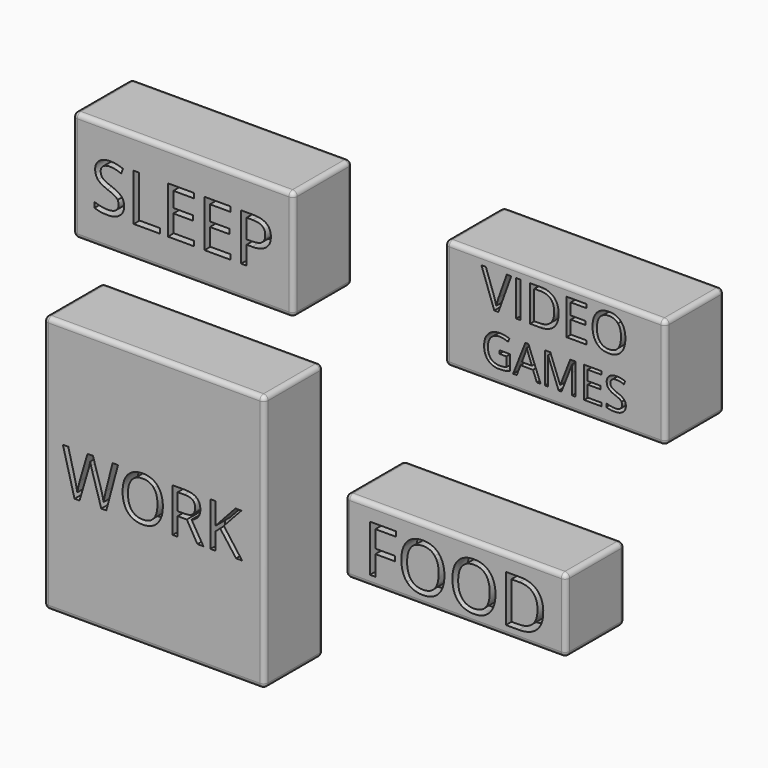
from build123d import *

# Parameters (mm, degrees)
F0_W           = 76.2
F0_H           = 88.9
F0_H_2         = 38.1
F0_W_2         = 1.4327720826
F0_H_3         = 12.3283157168
F0_H_4         = 25.4
F0_TEXT_SIZE   = 21.1578508955
F0_TEXT_SIZE_2 = 22.6268025166
F0_TEXT_SIZE_3 = 22.7127927122
F0_TEXT_SIZE_4 = 15.0053076107
F0_TEXT_SIZE_5 = 17.268816062
F1_DEPTH       = 19.05
F2_DEPTH       = 6.35
F3_R           = 1.5875


# Not quite as in the source:
# - Text() gives the source's letters only with a copy of the font that has no kerning and outlines rounded to 1/6400 em; it was checked with that copy


with BuildPart() as f1:
    # F0 (on Front) → F1 (new body)
    with BuildSketch(Plane.XZ):
        with Locations((-47.0108405503, -38.8578269625)):
            Rectangle(F0_W, F0_H)
        with BuildLine():
            Line((-59.4609134366, -31.3667576164), (-63.5007405919, -46.4714796072))
            Line((-63.5007405919, -46.4714796072), (-65.2363455482, -46.4714796072))
            Line((-65.2363455482, -46.4714796072), (-68.2843984428, -36.3586880621))
            add(Edge.make_bspline(
                [(-68.2843984428, -36.3586880621), (-68.5025887802, -35.6842815648), (-68.7703678306, -34.6627540762)],
                knots=[0, 0, 0, 1, 1, 1], degree=2))
            add(Edge.make_bspline(
                [(-68.7703678306, -34.6627540762), (-69.038146881, -33.6412265877), (-69.0480646236, -33.4329539929)],
                knots=[0, 0, 0, 1, 1, 1], degree=2))
            add(Edge.make_bspline(
                [(-69.0480646236, -33.4329539929), (-69.2761727036, -34.7982965585), (-69.7720598339, -36.4181945177)],
                knots=[0, 0, 0, 1, 1, 1], degree=2))
            Line((-69.7720598339, -36.4181945177), (-72.7275471309, -46.4714796072))
            Line((-72.7275471309, -46.4714796072), (-74.4631520871, -46.4714796072))
            Line((-74.4631520871, -46.4714796072), (-78.4831437573, -31.3667576164))
            Line((-78.4831437573, -31.3667576164), (-76.6219140613, -31.3667576164))
            Line((-76.6219140613, -31.3667576164), (-74.2350440072, -40.6960474956))
            add(Edge.make_bspline(
                [(-74.2350440072, -40.6960474956), (-73.7391568768, -42.6597605319), (-73.5110487968, -44.2499052632)],
                knots=[0, 0, 0, 1, 1, 1], degree=2))
            add(Edge.make_bspline(
                [(-73.5110487968, -44.2499052632), (-73.2333520038, -42.3589223394), (-72.6845702462, -40.5505872707)],
                knots=[0, 0, 0, 1, 1, 1], degree=2))
            Line((-72.6845702462, -40.5505872707), (-69.9803324287, -31.3667576164))
            Line((-69.9803324287, -31.3667576164), (-68.1191027327, -31.3667576164))
            Line((-68.1191027327, -31.3667576164), (-65.2793224328, -40.6332351258))
            add(Edge.make_bspline(
                [(-65.2793224328, -40.6332351258), (-64.7834353025, -42.2366035139), (-64.4429261396, -44.2499052632)],
                knots=[0, 0, 0, 1, 1, 1], degree=2))
            add(Edge.make_bspline(
                [(-64.4429261396, -44.2499052632), (-64.2445712875, -42.7820793573), (-63.6990954441, -40.6762120104)],
                knots=[0, 0, 0, 1, 1, 1], degree=2))
            Line((-63.6990954441, -40.6762120104), (-61.3221431325, -31.3667576164))
            Line((-61.3221431325, -31.3667576164), (-59.4609134366, -31.3667576164))
        make_face(mode=Mode.SUBTRACT)
        with BuildLine():
            add(Edge.make_bspline(
                [(-45.814099609, -33.1949281703), (-43.9859290551, -35.2611245469), (-43.9859290551, -38.8976301695)],
                knots=[0, 0, 0, 1, 1, 1], degree=2))
            add(Edge.make_bspline(
                [(-43.9859290551, -38.8976301695), (-43.9859290551, -42.5242180496), (-45.8207114374, -44.6019851258)],
                knots=[0, 0, 0, 1, 1, 1], degree=2))
            add(Edge.make_bspline(
                [(-45.8207114374, -44.6019851258), (-47.6554938198, -46.679752202), (-50.9184311375, -46.679752202)],
                knots=[0, 0, 0, 1, 1, 1], degree=2))
            add(Edge.make_bspline(
                [(-50.9184311375, -46.679752202), (-54.2540985678, -46.679752202), (-56.0673925078, -44.638350182)],
                knots=[0, 0, 0, 1, 1, 1], degree=2))
            add(Edge.make_bspline(
                [(-56.0673925078, -44.638350182), (-57.8806864478, -42.596948162), (-57.8806864478, -38.8777946843)],
                knots=[0, 0, 0, 1, 1, 1], degree=2))
            add(Edge.make_bspline(
                [(-57.8806864478, -38.8777946843), (-57.8806864478, -35.1883944344), (-56.0624336365, -33.1585631141)],
                knots=[0, 0, 0, 1, 1, 1], degree=2))
            add(Edge.make_bspline(
                [(-56.0624336365, -33.1585631141), (-54.2441808252, -31.1287317938), (-50.8985956523, -31.1287317938)],
                knots=[0, 0, 0, 1, 1, 1], degree=2))
            add(Edge.make_bspline(
                [(-50.8985956523, -31.1287317938), (-47.6422701629, -31.1287317938), (-45.814099609, -33.1949281703)],
                knots=[0, 0, 0, 1, 1, 1], degree=2))
        make_face(mode=Mode.SUBTRACT)
        with BuildLine():
            Line((-35.7112258064, -40.1902426227), (-38.8650679555, -40.1902426227))
            Line((-38.8650679555, -40.1902426227), (-38.8650679555, -46.4714796072))
            Line((-38.8650679555, -46.4714796072), (-40.620508397, -46.4714796072))
            Line((-40.620508397, -46.4714796072), (-40.620508397, -31.3667576164))
            Line((-40.620508397, -31.3667576164), (-36.4781979014, -31.3667576164))
            add(Edge.make_bspline(
                [(-36.4781979014, -31.3667576164), (-33.6979240572, -31.3667576164), (-32.3705995049, -32.4312619896)],
                knots=[0, 0, 0, 1, 1, 1], degree=2))
            add(Edge.make_bspline(
                [(-32.3705995049, -32.4312619896), (-31.0432749526, -33.4957663628), (-31.0432749526, -35.6346928517)],
                knots=[0, 0, 0, 1, 1, 1], degree=2))
            add(Edge.make_bspline(
                [(-31.0432749526, -35.6346928517), (-31.0432749526, -38.6298511191), (-34.0814101046, -39.6844377497)],
                knots=[0, 0, 0, 1, 1, 1], degree=2))
            Line((-34.0814101046, -39.6844377497), (-29.9787705794, -46.4714796072))
            Line((-29.9787705794, -46.4714796072), (-32.0548846986, -46.4714796072))
            Line((-32.0548846986, -46.4714796072), (-35.7112258064, -40.1902426227))
        make_face(mode=Mode.SUBTRACT)
        Polygon((-22.9338674141, -37.9289973082), (-16.6327949443, -46.4714796072), (-18.6989913208, -46.4714796072), (-24.2033384678, -39.1455737347), (-25.7868713708, -40.5505872707), (-25.7868713708, -46.4714796072), (-27.5423118123, -46.4714796072), (-27.5423118123, -31.3667576164), (-25.7868713708, -31.3667576164), (-25.7868713708, -38.8579591991), (-18.9370171434, -31.3667576164), (-16.8609030243, -31.3667576164), align=None, mode=Mode.SUBTRACT)
        with Locations((-36.9797299606, 51.8156976043)):
            Rectangle(F0_W, F0_H_2)
        with BuildLine():
            add(Edge.make_bspline(
                [(-58.3102363038, 50.6565701019), (-57.3520403613, 49.6132011867), (-57.3520403613, 47.9523282196)],
                knots=[0, 0, 0, 1, 1, 1], degree=2))
            add(Edge.make_bspline(
                [(-57.3520403613, 47.9523282196), (-57.3520403613, 45.8123572812), (-58.9046726756, 44.6128379161)],
                knots=[0, 0, 0, 1, 1, 1], degree=2))
            add(Edge.make_bspline(
                [(-58.9046726756, 44.6128379161), (-60.4573049899, 43.413318551), (-63.1189603859, 43.413318551)],
                knots=[0, 0, 0, 1, 1, 1], degree=2))
            add(Edge.make_bspline(
                [(-63.1189603859, 43.413318551), (-66.0006459612, 43.413318551), (-67.5550527125, 44.1585820619)],
                knots=[0, 0, 0, 1, 1, 1], degree=2))
            Line((-67.5550527125, 44.1585820619), (-67.5550527125, 45.9756054789))
            add(Edge.make_bspline(
                [(-67.5550527125, 45.9756054789), (-66.5542702836, 45.5568383632), (-65.3795930355, 45.3119660668)],
                knots=[0, 0, 0, 1, 1, 1], degree=2))
            add(Edge.make_bspline(
                [(-65.3795930355, 45.3119660668), (-64.2049157874, 45.0670937704), (-63.0515317825, 45.0670937704)],
                knots=[0, 0, 0, 1, 1, 1], degree=2))
            add(Edge.make_bspline(
                [(-63.0515317825, 45.0670937704), (-61.1670797622, 45.0670937704), (-60.2124326935, 45.7821918534)],
                knots=[0, 0, 0, 1, 1, 1], degree=2))
            add(Edge.make_bspline(
                [(-60.2124326935, 45.7821918534), (-59.2577856248, 46.4972899365), (-59.2577856248, 47.7748845265)],
                knots=[0, 0, 0, 1, 1, 1], degree=2))
            add(Edge.make_bspline(
                [(-59.2577856248, 47.7748845265), (-59.2577856248, 48.6159676317), (-59.5967030786, 49.1536220216)],
                knots=[0, 0, 0, 1, 1, 1], degree=2))
            add(Edge.make_bspline(
                [(-59.5967030786, 49.1536220216), (-59.9356205323, 49.6912764116), (-60.7287938403, 50.1473067028)],
                knots=[0, 0, 0, 1, 1, 1], degree=2))
            add(Edge.make_bspline(
                [(-60.7287938403, 50.1473067028), (-61.5219671483, 50.603336994), (-63.1402536291, 51.1782545595)],
                knots=[0, 0, 0, 1, 1, 1], degree=2))
            add(Edge.make_bspline(
                [(-63.1402536291, 51.1782545595), (-65.4008862787, 51.9873977999), (-66.3715032798, 53.0964208815)],
                knots=[0, 0, 0, 1, 1, 1], degree=2))
            add(Edge.make_bspline(
                [(-66.3715032798, 53.0964208815), (-67.3421202808, 54.2054439632), (-67.3421202808, 55.9905275154)],
                knots=[0, 0, 0, 1, 1, 1], degree=2))
            add(Edge.make_bspline(
                [(-67.3421202808, 55.9905275154), (-67.3421202808, 57.8643329142), (-65.9349917948, 58.9733559958)],
                knots=[0, 0, 0, 1, 1, 1], degree=2))
            add(Edge.make_bspline(
                [(-65.9349917948, 58.9733559958), (-64.5278633088, 60.0823790775), (-62.2068998035, 60.0823790775)],
                knots=[0, 0, 0, 1, 1, 1], degree=2))
            add(Edge.make_bspline(
                [(-62.2068998035, 60.0823790775), (-59.790116704, 60.0823790775), (-57.7601608553, 59.1951606122)],
                knots=[0, 0, 0, 1, 1, 1], degree=2))
            Line((-57.7601608553, 59.1951606122), (-58.3492739163, 57.5555808882))
            add(Edge.make_bspline(
                [(-58.3492739163, 57.5555808882), (-60.3579365218, 58.3966639934), (-62.2530351637, 58.3966639934)],
                knots=[0, 0, 0, 1, 1, 1], degree=2))
            add(Edge.make_bspline(
                [(-62.2530351637, 58.3966639934), (-63.7506599332, 58.3966639934), (-64.5935174752, 57.7543178245)],
                knots=[0, 0, 0, 1, 1, 1], degree=2))
            add(Edge.make_bspline(
                [(-64.5935174752, 57.7543178245), (-65.4363750173, 57.1119716556), (-65.4363750173, 55.9692342722)],
                knots=[0, 0, 0, 1, 1, 1], degree=2))
            add(Edge.make_bspline(
                [(-65.4363750173, 55.9692342722), (-65.4363750173, 55.1281511671), (-65.1258485544, 54.5887223402)],
                knots=[0, 0, 0, 1, 1, 1], degree=2))
            add(Edge.make_bspline(
                [(-65.1258485544, 54.5887223402), (-64.8153220916, 54.0492935133), (-64.0771563284, 53.6003609698)],
                knots=[0, 0, 0, 1, 1, 1], degree=2))
            add(Edge.make_bspline(
                [(-64.0771563284, 53.6003609698), (-63.3389905653, 53.1514284264), (-61.8200725527, 52.6084507256)],
                knots=[0, 0, 0, 1, 1, 1], degree=2))
            add(Edge.make_bspline(
                [(-61.8200725527, 52.6084507256), (-59.2684322464, 51.6999390171), (-58.3102363038, 50.6565701019)],
                knots=[0, 0, 0, 1, 1, 1], degree=2))
        make_face(mode=Mode.SUBTRACT)
        Polygon((-44.9948615763, 43.6368976043), (-54.033843301, 43.6368976043), (-54.033843301, 59.8517022765), (-52.1493912806, 59.8517022765), (-52.1493912806, 45.3439059316), (-44.9948615763, 45.3439059316), align=None, mode=Mode.SUBTRACT)
        Polygon((-33.2055026091, 45.3226126884), (-33.2055026091, 43.6368976043), (-42.2444843338, 43.6368976043), (-42.2444843338, 59.8517022765), (-33.2055026091, 59.8517022765), (-33.2055026091, 58.176633814), (-40.3600323135, 58.176633814), (-40.3600323135, 52.9526914901), (-33.6384652202, 52.9526914901), (-33.6384652202, 51.2882696492), (-40.3600323135, 51.2882696492), (-40.3600323135, 45.3226126884), align=None, mode=Mode.SUBTRACT)
        Polygon((-20.5750605368, 45.3226126884), (-20.5750605368, 43.6368976043), (-29.6140422615, 43.6368976043), (-29.6140422615, 59.8517022765), (-20.5750605368, 59.8517022765), (-20.5750605368, 58.176633814), (-27.7295902411, 58.176633814), (-27.7295902411, 52.9526914901), (-21.0080231479, 52.9526914901), (-21.0080231479, 51.2882696492), (-27.7295902411, 51.2882696492), (-27.7295902411, 45.3226126884), align=None, mode=Mode.SUBTRACT)
        with BuildLine():
            add(Edge.make_bspline(
                [(-12.7781846635, 59.8517022765), (-6.702512613, 59.8517022765), (-6.702512613, 55.1281511671)],
                knots=[0, 0, 0, 1, 1, 1], degree=2))
            add(Edge.make_bspline(
                [(-6.702512613, 55.1281511671), (-6.702512613, 52.6652327074), (-8.3829043863, 51.3397283202)],
                knots=[0, 0, 0, 1, 1, 1], degree=2))
            add(Edge.make_bspline(
                [(-8.3829043863, 51.3397283202), (-10.0632961596, 50.014223933), (-13.1898540314, 50.014223933)],
                knots=[0, 0, 0, 1, 1, 1], degree=2))
            Line((-13.1898540314, 50.014223933), (-15.0991481688, 50.014223933))
            Line((-15.0991481688, 50.014223933), (-15.0991481688, 43.6368976043))
            Line((-15.0991481688, 43.6368976043), (-16.9836001892, 43.6368976043))
            Line((-16.9836001892, 43.6368976043), (-16.9836001892, 59.8517022765))
            Line((-16.9836001892, 59.8517022765), (-12.7781846635, 59.8517022765))
        make_face(mode=Mode.SUBTRACT)
        with Locations((91.3764792442, 54.6455720641)):
            Rectangle(F0_W, F0_H_2)
        with BuildLine():
            Line((72.161479475, 45.2315640381), (72.161479475, 46.3452392123))
            Line((72.161479475, 46.3452392123), (75.8026111499, 46.3452392123))
            Line((75.8026111499, 46.3452392123), (75.8026111499, 41.1355839762))
            add(Edge.make_bspline(
                [(75.8026111499, 41.1355839762), (74.9515288589, 40.8636127758), (74.072311616, 40.7241103066)],
                knots=[0, 0, 0, 1, 1, 1], degree=2))
            add(Edge.make_bspline(
                [(74.072311616, 40.7241103066), (73.1930943732, 40.5846078374), (72.034872192, 40.5846078374)],
                knots=[0, 0, 0, 1, 1, 1], degree=2))
            add(Edge.make_bspline(
                [(72.034872192, 40.5846078374), (69.6035434432, 40.5846078374), (68.2483765997, 42.0323855639)],
                knots=[0, 0, 0, 1, 1, 1], degree=2))
            add(Edge.make_bspline(
                [(68.2483765997, 42.0323855639), (66.8932097561, 43.4801632904), (66.8932097561, 46.0873354877)],
                knots=[0, 0, 0, 1, 1, 1], degree=2))
            add(Edge.make_bspline(
                [(66.8932097561, 46.0873354877), (66.8932097561, 47.7590205387), (67.5637594399, 49.0157150511)],
                knots=[0, 0, 0, 1, 1, 1], degree=2))
            add(Edge.make_bspline(
                [(67.5637594399, 49.0157150511), (68.2343091238, 50.2724095635), (69.4945205051, 50.9347532198)],
                knots=[0, 0, 0, 1, 1, 1], degree=2))
            add(Edge.make_bspline(
                [(69.4945205051, 50.9347532198), (70.7547318865, 51.597096876), (72.445173572, 51.597096876)],
                knots=[0, 0, 0, 1, 1, 1], degree=2))
            add(Edge.make_bspline(
                [(72.445173572, 51.597096876), (74.16140563, 51.597096876), (75.6408351772, 50.9687496198)],
                knots=[0, 0, 0, 1, 1, 1], degree=2))
            Line((75.6408351772, 50.9687496198), (75.1578518385, 49.8691419215))
            add(Edge.make_bspline(
                [(75.1578518385, 49.8691419215), (73.706557243, 50.4834217018), (72.3654578753, 50.4834217018)],
                knots=[0, 0, 0, 1, 1, 1], degree=2))
            add(Edge.make_bspline(
                [(72.3654578753, 50.4834217018), (70.4100787273, 50.4834217018), (69.310471029, 49.3193380723)],
                knots=[0, 0, 0, 1, 1, 1], degree=2))
            add(Edge.make_bspline(
                [(69.310471029, 49.3193380723), (68.2108633306, 48.1552544428), (68.2108633306, 46.0873354877)],
                knots=[0, 0, 0, 1, 1, 1], degree=2))
            add(Edge.make_bspline(
                [(68.2108633306, 46.0873354877), (68.2108633306, 43.9185996221), (69.269440891, 42.79789071)],
                knots=[0, 0, 0, 1, 1, 1], degree=2))
            add(Edge.make_bspline(
                [(69.269440891, 42.79789071), (70.3280184513, 41.6771817978), (72.3795253512, 41.6771817978)],
                knots=[0, 0, 0, 1, 1, 1], degree=2))
            add(Edge.make_bspline(
                [(72.3795253512, 41.6771817978), (73.4932005254, 41.6771817978), (74.5552949548, 41.9350855223)],
                knots=[0, 0, 0, 1, 1, 1], degree=2))
            Line((74.5552949548, 41.9350855223), (74.5552949548, 45.2315640381))
            Line((74.5552949548, 45.2315640381), (72.161479475, 45.2315640381))
        make_face(mode=Mode.SUBTRACT)
        with BuildLine():
            Line((71.8964452505, 62.2214219074), (74.7134208706, 70.1488877809))
            Line((74.7134208706, 70.1488877809), (76.2541230537, 70.1488877809))
            Line((76.2541230537, 70.1488877809), (71.8127994227, 57.8205720641))
            Line((71.8127994227, 57.8205720641), (70.3962168551, 57.8205720641))
            Line((70.3962168551, 57.8205720641), (65.9764792442, 70.1488877809))
            Line((65.9764792442, 70.1488877809), (67.4955954072, 70.1488877809))
            Line((67.4955954072, 70.1488877809), (70.3287605424, 62.1728533623))
            add(Edge.make_bspline(
                [(70.3287605424, 62.1728533623), (70.8171442466, 60.7967445823), (71.1031590126, 59.4988851251)],
                knots=[0, 0, 0, 1, 1, 1], degree=2))
            add(Edge.make_bspline(
                [(71.1031590126, 59.4988851251), (71.4080615462, 60.8642008951), (71.8964452505, 62.2214219074)],
                knots=[0, 0, 0, 1, 1, 1], degree=2))
        make_face(mode=Mode.SUBTRACT)
        Polygon((86.3954204913, 40.7323163342), (85.1059018685, 40.7323163342), (83.7718362387, 44.1389900777), (79.4789115145, 44.1389900777), (78.1612579399, 40.7323163342), (76.8998742689, 40.7323163342), (81.1341845103, 51.4892462276), (82.1822114637, 51.4892462276), align=None, mode=Mode.SUBTRACT)
        with BuildLine():
            Line((93.6120356203, 40.7323163342), (92.6085556738, 40.7323163342))
            Line((92.6085556738, 40.7323163342), (88.9744577369, 50.2278625565))
            Line((88.9744577369, 50.2278625565), (88.915843254, 50.2278625565))
            add(Edge.make_bspline(
                [(88.915843254, 50.2278625565), (89.0190047438, 49.1001199064), (89.0190047438, 47.5456638211)],
                knots=[0, 0, 0, 1, 1, 1], degree=2))
            Line((89.0190047438, 47.5456638211), (89.0190047438, 40.7323163342))
            Line((89.0190047438, 40.7323163342), (87.8678163006, 40.7323163342))
            Line((87.8678163006, 40.7323163342), (87.8678163006, 51.4446992206))
            Line((87.8678163006, 51.4446992206), (89.7434797519, 51.4446992206))
            Line((89.7434797519, 51.4446992206), (93.1360860195, 42.6079797855))
            Line((93.1360860195, 42.6079797855), (93.1947005024, 42.6079797855))
            Line((93.1947005024, 42.6079797855), (96.6154417217, 51.4446992206))
            Line((96.6154417217, 51.4446992206), (98.4770376972, 51.4446992206))
            Line((98.4770376972, 51.4446992206), (98.4770376972, 40.7323163342))
            Line((98.4770376972, 40.7323163342), (97.2320660814, 40.7323163342))
            Line((97.2320660814, 40.7323163342), (97.2320660814, 47.6347578351))
            add(Edge.make_bspline(
                [(97.2320660814, 47.6347578351), (97.2320660814, 48.821114968), (97.3352275712, 50.2137950807)],
                knots=[0, 0, 0, 1, 1, 1], degree=2))
            Line((97.3352275712, 50.2137950807), (97.2766130883, 50.2137950807))
            Line((97.2766130883, 50.2137950807), (93.6120356203, 40.7323163342))
        make_face(mode=Mode.SUBTRACT)
        Polygon((107.386439091, 41.8459915084), (107.386439091, 40.7323163342), (101.4147955778, 40.7323163342), (101.4147955778, 51.4446992206), (107.386439091, 51.4446992206), (107.386439091, 50.3380577843), (102.6597671936, 50.3380577843), (102.6597671936, 46.8868370339), (107.1004004147, 46.8868370339), (107.1004004147, 45.7872293355), (102.6597671936, 45.7872293355), (102.6597671936, 41.8459915084), align=None, mode=Mode.SUBTRACT)
        with BuildLine():
            add(Edge.make_bspline(
                [(115.170442414, 45.3698942176), (115.8034788289, 44.6805878992), (115.8034788289, 43.5833247802)],
                knots=[0, 0, 0, 1, 1, 1], degree=2))
            add(Edge.make_bspline(
                [(115.8034788289, 43.5833247802), (115.8034788289, 42.1695434538), (114.7777253789, 41.3770756456)],
                knots=[0, 0, 0, 1, 1, 1], degree=2))
            add(Edge.make_bspline(
                [(114.7777253789, 41.3770756456), (113.751971929, 40.5846078374), (111.9935374433, 40.5846078374)],
                knots=[0, 0, 0, 1, 1, 1], degree=2))
            add(Edge.make_bspline(
                [(111.9935374433, 40.5846078374), (110.0897390402, 40.5846078374), (109.0628133006, 41.0769694934)],
                knots=[0, 0, 0, 1, 1, 1], degree=2))
            Line((109.0628133006, 41.0769694934), (109.0628133006, 42.2773941022))
            add(Edge.make_bspline(
                [(109.0628133006, 42.2773941022), (109.7239846672, 42.0007337431), (110.5000404202, 41.8389577705)],
                knots=[0, 0, 0, 1, 1, 1], degree=2))
            add(Edge.make_bspline(
                [(110.5000404202, 41.8389577705), (111.2760961732, 41.6771817978), (112.0380844503, 41.6771817978)],
                knots=[0, 0, 0, 1, 1, 1], degree=2))
            add(Edge.make_bspline(
                [(112.0380844503, 41.6771817978), (113.2830560661, 41.6771817978), (113.9137479016, 42.1496145296)],
                knots=[0, 0, 0, 1, 1, 1], degree=2))
            add(Edge.make_bspline(
                [(113.9137479016, 42.1496145296), (114.5444397371, 42.6220472614), (114.5444397371, 43.4660958145)],
                knots=[0, 0, 0, 1, 1, 1], degree=2))
            add(Edge.make_bspline(
                [(114.5444397371, 43.4660958145), (114.5444397371, 44.021761112), (114.3205324126, 44.376964878)],
                knots=[0, 0, 0, 1, 1, 1], degree=2))
            add(Edge.make_bspline(
                [(114.3205324126, 44.376964878), (114.0966250881, 44.7321686441), (113.5726116114, 45.033447086)],
                knots=[0, 0, 0, 1, 1, 1], degree=2))
            add(Edge.make_bspline(
                [(113.5726116114, 45.033447086), (113.0485981347, 45.3347255279), (111.9794699675, 45.7145473768)],
                knots=[0, 0, 0, 1, 1, 1], degree=2))
            add(Edge.make_bspline(
                [(111.9794699675, 45.7145473768), (110.4859729443, 46.2491114604), (109.8447305019, 46.9817924961)],
                knots=[0, 0, 0, 1, 1, 1], degree=2))
            add(Edge.make_bspline(
                [(109.8447305019, 46.9817924961), (109.2034880595, 47.7144735318), (109.2034880595, 48.8937969268)],
                knots=[0, 0, 0, 1, 1, 1], degree=2))
            add(Edge.make_bspline(
                [(109.2034880595, 48.8937969268), (109.2034880595, 50.1317348047), (110.1331137575, 50.8644158403)],
                knots=[0, 0, 0, 1, 1, 1], degree=2))
            add(Edge.make_bspline(
                [(110.1331137575, 50.8644158403), (111.0627394556, 51.597096876), (112.5960943271, 51.597096876)],
                knots=[0, 0, 0, 1, 1, 1], degree=2))
            add(Edge.make_bspline(
                [(112.5960943271, 51.597096876), (114.19275284, 51.597096876), (115.5338522077, 51.0109520475)],
                knots=[0, 0, 0, 1, 1, 1], degree=2))
            Line((115.5338522077, 51.0109520475), (115.1446520416, 49.9277564043))
            add(Edge.make_bspline(
                [(115.1446520416, 49.9277564043), (113.8176201498, 50.4834217018), (112.565614796, 50.4834217018)],
                knots=[0, 0, 0, 1, 1, 1], degree=2))
            add(Edge.make_bspline(
                [(112.565614796, 50.4834217018), (111.5762023254, 50.4834217018), (111.0193647383, 50.0590528459)],
                knots=[0, 0, 0, 1, 1, 1], degree=2))
            add(Edge.make_bspline(
                [(111.0193647383, 50.0590528459), (110.4625271512, 49.6346839901), (110.4625271512, 48.8797294509)],
                knots=[0, 0, 0, 1, 1, 1], degree=2))
            add(Edge.make_bspline(
                [(110.4625271512, 48.8797294509), (110.4625271512, 48.3240641534), (110.6676778412, 47.9676880977)],
                knots=[0, 0, 0, 1, 1, 1], degree=2))
            add(Edge.make_bspline(
                [(110.6676778412, 47.9676880977), (110.8728285312, 47.6113120419), (111.3605010285, 47.3147227587)],
                knots=[0, 0, 0, 1, 1, 1], degree=2))
            add(Edge.make_bspline(
                [(111.3605010285, 47.3147227587), (111.8481735259, 47.0181334755), (112.8516534723, 46.6594128404)],
                knots=[0, 0, 0, 1, 1, 1], degree=2))
            add(Edge.make_bspline(
                [(112.8516534723, 46.6594128404), (114.5374059992, 46.059200536), (115.170442414, 45.3698942176)],
                knots=[0, 0, 0, 1, 1, 1], degree=2))
        make_face(mode=Mode.SUBTRACT)
        with Locations((78.6650116711, 63.9847299225)):
            Rectangle(F0_W_2, F0_H_3, mode=Mode.SUBTRACT)
        with BuildLine():
            add(Edge.make_bspline(
                [(91.0095169029, 68.5555696739), (92.6028350099, 66.962251567), (92.6028350099, 64.1021039067)],
                knots=[0, 0, 0, 1, 1, 1], degree=2))
            add(Edge.make_bspline(
                [(92.6028350099, 64.1021039067), (92.6028350099, 61.0503803182), (90.9461079689, 59.4354761912)],
                knots=[0, 0, 0, 1, 1, 1], degree=2))
            add(Edge.make_bspline(
                [(90.9461079689, 59.4354761912), (89.289380928, 57.8205720641), (86.1782957843, 57.8205720641)],
                knots=[0, 0, 0, 1, 1, 1], degree=2))
            Line((86.1782957843, 57.8205720641), (82.762308107, 57.8205720641))
            Line((82.762308107, 57.8205720641), (82.762308107, 70.1488877809))
            Line((82.762308107, 70.1488877809), (86.5398616206, 70.1488877809))
            add(Edge.make_bspline(
                [(86.5398616206, 70.1488877809), (89.4161987959, 70.1488877809), (91.0095169029, 68.5555696739)],
                knots=[0, 0, 0, 1, 1, 1], degree=2))
        make_face(mode=Mode.SUBTRACT)
        Polygon((102.2248034595, 59.1022420062), (102.2248034595, 57.8205720641), (95.3523543173, 57.8205720641), (95.3523543173, 70.1488877809), (102.2248034595, 70.1488877809), (102.2248034595, 68.8753125963), (96.7851263999, 68.8753125963), (96.7851263999, 64.9034849021), (101.8956166533, 64.9034849021), (101.8956166533, 63.638004475), (96.7851263999, 63.638004475), (96.7851263999, 59.1022420062), align=None, mode=Mode.SUBTRACT)
        with BuildLine():
            add(Edge.make_bspline(
                [(114.1645708148, 68.656754143), (115.6567044527, 66.9703463245), (115.6567044527, 64.0022685638)],
                knots=[0, 0, 0, 1, 1, 1], degree=2))
            add(Edge.make_bspline(
                [(115.6567044527, 64.0022685638), (115.6567044527, 61.0422855607), (114.1591743098, 59.3464338584)],
                knots=[0, 0, 0, 1, 1, 1], degree=2))
            add(Edge.make_bspline(
                [(114.1591743098, 59.3464338584), (112.6616441669, 57.650582156), (109.9984689399, 57.650582156)],
                knots=[0, 0, 0, 1, 1, 1], degree=2))
            add(Edge.make_bspline(
                [(109.9984689399, 57.650582156), (107.2759321576, 57.650582156), (105.795940656, 59.3167530807)],
                knots=[0, 0, 0, 1, 1, 1], degree=2))
            add(Edge.make_bspline(
                [(105.795940656, 59.3167530807), (104.3159491545, 60.9829240055), (104.3159491545, 64.0184580789)],
                knots=[0, 0, 0, 1, 1, 1], degree=2))
            add(Edge.make_bspline(
                [(104.3159491545, 64.0184580789), (104.3159491545, 67.0297078797), (105.7999880348, 68.6864349207)],
                knots=[0, 0, 0, 1, 1, 1], degree=2))
            add(Edge.make_bspline(
                [(105.7999880348, 68.6864349207), (107.2840269151, 70.3431619616), (110.0146584549, 70.3431619616)],
                knots=[0, 0, 0, 1, 1, 1], degree=2))
            add(Edge.make_bspline(
                [(110.0146584549, 70.3431619616), (112.672437177, 70.3431619616), (114.1645708148, 68.656754143)],
                knots=[0, 0, 0, 1, 1, 1], degree=2))
        make_face(mode=Mode.SUBTRACT)
        with Locations((57.0269852698, -27.2473629941)):
            Rectangle(F0_W, F0_H_4)
        Polygon((29.374557788, -29.531857243), (29.374557788, -36.4365674485), (27.4972402667, -36.4365674485), (27.4972402667, -20.2831517144), (36.5020005807, -20.2831517144), (36.5020005807, -21.9518784), (29.374557788, -21.9518784), (29.374557788, -27.8631305574), (36.0706771578, -27.8631305574), (36.0706771578, -29.531857243), align=None, mode=Mode.SUBTRACT)
        with BuildLine():
            add(Edge.make_bspline(
                [(51.2412411575, -22.2382488693), (53.1963383125, -24.4478975526), (53.1963383125, -28.3368792351)],
                knots=[0, 0, 0, 1, 1, 1], degree=2))
            add(Edge.make_bspline(
                [(53.1963383125, -28.3368792351), (53.1963383125, -32.215254604), (51.2341702818, -34.4372773199)],
                knots=[0, 0, 0, 1, 1, 1], degree=2))
            add(Edge.make_bspline(
                [(51.2341702818, -34.4372773199), (49.272002251, -36.6593000358), (45.7825250504, -36.6593000358)],
                knots=[0, 0, 0, 1, 1, 1], degree=2))
            add(Edge.make_bspline(
                [(45.7825250504, -36.6593000358), (42.2152682162, -36.6593000358), (40.2760805317, -34.4761671367)],
                knots=[0, 0, 0, 1, 1, 1], degree=2))
            add(Edge.make_bspline(
                [(40.2760805317, -34.4761671367), (38.3368928473, -32.2930342376), (38.3368928473, -28.3156666078)],
                knots=[0, 0, 0, 1, 1, 1], degree=2))
            add(Edge.make_bspline(
                [(38.3368928473, -28.3156666078), (38.3368928473, -24.370117919), (40.2813836886, -22.1993590525)],
                knots=[0, 0, 0, 1, 1, 1], degree=2))
            add(Edge.make_bspline(
                [(40.2813836886, -22.1993590525), (42.2258745298, -20.0286001861), (45.8037376778, -20.0286001861)],
                knots=[0, 0, 0, 1, 1, 1], degree=2))
            add(Edge.make_bspline(
                [(45.8037376778, -20.0286001861), (49.2861440026, -20.0286001861), (51.2412411575, -22.2382488693)],
                knots=[0, 0, 0, 1, 1, 1], degree=2))
        make_face(mode=Mode.SUBTRACT)
        with BuildLine():
            add(Edge.make_bspline(
                [(68.8618636173, -22.2382488693), (70.8169607723, -24.4478975526), (70.8169607723, -28.3368792351)],
                knots=[0, 0, 0, 1, 1, 1], degree=2))
            add(Edge.make_bspline(
                [(70.8169607723, -28.3368792351), (70.8169607723, -32.215254604), (68.8547927415, -34.4372773199)],
                knots=[0, 0, 0, 1, 1, 1], degree=2))
            add(Edge.make_bspline(
                [(68.8547927415, -34.4372773199), (66.8926247108, -36.6593000358), (63.4031475102, -36.6593000358)],
                knots=[0, 0, 0, 1, 1, 1], degree=2))
            add(Edge.make_bspline(
                [(63.4031475102, -36.6593000358), (59.8358906759, -36.6593000358), (57.8967029915, -34.4761671367)],
                knots=[0, 0, 0, 1, 1, 1], degree=2))
            add(Edge.make_bspline(
                [(57.8967029915, -34.4761671367), (55.9575153071, -32.2930342376), (55.9575153071, -28.3156666078)],
                knots=[0, 0, 0, 1, 1, 1], degree=2))
            add(Edge.make_bspline(
                [(55.9575153071, -28.3156666078), (55.9575153071, -24.370117919), (57.9020061484, -22.1993590525)],
                knots=[0, 0, 0, 1, 1, 1], degree=2))
            add(Edge.make_bspline(
                [(57.9020061484, -22.1993590525), (59.8464969896, -20.0286001861), (63.4243601376, -20.0286001861)],
                knots=[0, 0, 0, 1, 1, 1], degree=2))
            add(Edge.make_bspline(
                [(63.4243601376, -20.0286001861), (66.9067664624, -20.0286001861), (68.8618636173, -22.2382488693)],
                knots=[0, 0, 0, 1, 1, 1], degree=2))
        make_face(mode=Mode.SUBTRACT)
        with BuildLine():
            add(Edge.make_bspline(
                [(85.2221024682, -22.3708277903), (87.3097785441, -24.4585038663), (87.3097785441, -28.2060680331)],
                knots=[0, 0, 0, 1, 1, 1], degree=2))
            add(Edge.make_bspline(
                [(87.3097785441, -28.2060680331), (87.3097785441, -32.2046482903), (85.1390196777, -34.3206078694)],
                knots=[0, 0, 0, 1, 1, 1], degree=2))
            add(Edge.make_bspline(
                [(85.1390196777, -34.3206078694), (82.9682608112, -36.4365674485), (78.8919009204, -36.4365674485)],
                knots=[0, 0, 0, 1, 1, 1], degree=2))
            Line((78.8919009204, -36.4365674485), (74.4160365476, -36.4365674485))
            Line((74.4160365476, -36.4365674485), (74.4160365476, -20.2831517144))
            Line((74.4160365476, -20.2831517144), (79.3656495981, -20.2831517144))
            add(Edge.make_bspline(
                [(79.3656495981, -20.2831517144), (83.1344263922, -20.2831517144), (85.2221024682, -22.3708277903)],
                knots=[0, 0, 0, 1, 1, 1], degree=2))
        make_face(mode=Mode.SUBTRACT)
        with BuildLine():
            add(Edge.make_bspline(
                [(41.7220746301, -23.4049433741), (40.3238089433, -25.1019535628), (40.3238089433, -28.3368792351)],
                knots=[0, 0, 0, 1, 1, 1], degree=2))
            add(Edge.make_bspline(
                [(40.3238089433, -28.3368792351), (40.3238089433, -31.6177656), (41.7220746301, -33.3147757888)],
                knots=[0, 0, 0, 1, 1, 1], degree=2))
            add(Edge.make_bspline(
                [(41.7220746301, -33.3147757888), (43.1203403168, -35.0117859775), (45.7825250504, -35.0117859775)],
                knots=[0, 0, 0, 1, 1, 1], degree=2))
            add(Edge.make_bspline(
                [(45.7825250504, -35.0117859775), (48.4659224114, -35.0117859775), (49.835904595, -33.3218466646)],
                knots=[0, 0, 0, 1, 1, 1], degree=2))
            add(Edge.make_bspline(
                [(49.835904595, -33.3218466646), (51.2058867786, -31.6319073516), (51.2058867786, -28.3368792351)],
                knots=[0, 0, 0, 1, 1, 1], degree=2))
            add(Edge.make_bspline(
                [(51.2058867786, -28.3368792351), (51.2058867786, -25.0772054976), (49.8412077518, -23.3925693415)],
                knots=[0, 0, 0, 1, 1, 1], degree=2))
            add(Edge.make_bspline(
                [(49.8412077518, -23.3925693415), (48.4765287251, -21.7079331854), (45.8037376778, -21.7079331854)],
                knots=[0, 0, 0, 1, 1, 1], degree=2))
            add(Edge.make_bspline(
                [(45.8037376778, -21.7079331854), (43.1203403168, -21.7079331854), (41.7220746301, -23.4049433741)],
                knots=[0, 0, 0, 1, 1, 1], degree=2))
        make_face()
        with BuildLine():
            add(Edge.make_bspline(
                [(59.3426970898, -23.4049433741), (57.9444314031, -25.1019535628), (57.9444314031, -28.3368792351)],
                knots=[0, 0, 0, 1, 1, 1], degree=2))
            add(Edge.make_bspline(
                [(57.9444314031, -28.3368792351), (57.9444314031, -31.6177656), (59.3426970898, -33.3147757888)],
                knots=[0, 0, 0, 1, 1, 1], degree=2))
            add(Edge.make_bspline(
                [(59.3426970898, -33.3147757888), (60.7409627766, -35.0117859775), (63.4031475102, -35.0117859775)],
                knots=[0, 0, 0, 1, 1, 1], degree=2))
            add(Edge.make_bspline(
                [(63.4031475102, -35.0117859775), (66.0865448711, -35.0117859775), (67.4565270548, -33.3218466646)],
                knots=[0, 0, 0, 1, 1, 1], degree=2))
            add(Edge.make_bspline(
                [(67.4565270548, -33.3218466646), (68.8265092384, -31.6319073516), (68.8265092384, -28.3368792351)],
                knots=[0, 0, 0, 1, 1, 1], degree=2))
            add(Edge.make_bspline(
                [(68.8265092384, -28.3368792351), (68.8265092384, -25.0772054976), (67.4618302116, -23.3925693415)],
                knots=[0, 0, 0, 1, 1, 1], degree=2))
            add(Edge.make_bspline(
                [(67.4618302116, -23.3925693415), (66.0971511848, -21.7079331854), (63.4243601376, -21.7079331854)],
                knots=[0, 0, 0, 1, 1, 1], degree=2))
            add(Edge.make_bspline(
                [(63.4243601376, -21.7079331854), (60.7409627766, -21.7079331854), (59.3426970898, -23.4049433741)],
                knots=[0, 0, 0, 1, 1, 1], degree=2))
        make_face()
        with BuildLine():
            add(Edge.make_bspline(
                [(-54.715273599, -34.2858798571), (-56.0227626661, -35.8727186743), (-56.0227626661, -38.8976301695)],
                knots=[0, 0, 0, 1, 1, 1], degree=2))
            add(Edge.make_bspline(
                [(-56.0227626661, -38.8976301695), (-56.0227626661, -41.9655185493), (-54.715273599, -43.5523573665)],
                knots=[0, 0, 0, 1, 1, 1], degree=2))
            add(Edge.make_bspline(
                [(-54.715273599, -43.5523573665), (-53.407784532, -45.1391961837), (-50.9184311375, -45.1391961837)],
                knots=[0, 0, 0, 1, 1, 1], degree=2))
            add(Edge.make_bspline(
                [(-50.9184311375, -45.1391961837), (-48.4092422579, -45.1391961837), (-47.1282005045, -43.5589691949)],
                knots=[0, 0, 0, 1, 1, 1], degree=2))
            add(Edge.make_bspline(
                [(-47.1282005045, -43.5589691949), (-45.847158751, -41.9787422062), (-45.847158751, -38.8976301695)],
                knots=[0, 0, 0, 1, 1, 1], degree=2))
            add(Edge.make_bspline(
                [(-45.847158751, -38.8976301695), (-45.847158751, -35.8495772749), (-47.1232416332, -34.2743091574)],
                knots=[0, 0, 0, 1, 1, 1], degree=2))
            add(Edge.make_bspline(
                [(-47.1232416332, -34.2743091574), (-48.3993245153, -32.69904104), (-50.8985956523, -32.69904104)],
                knots=[0, 0, 0, 1, 1, 1], degree=2))
            add(Edge.make_bspline(
                [(-50.8985956523, -32.69904104), (-53.407784532, -32.69904104), (-54.715273599, -34.2858798571)],
                knots=[0, 0, 0, 1, 1, 1], degree=2))
        make_face()
        with BuildLine():
            add(Edge.make_bspline(
                [(83.6311554162, -33.1609842404), (85.3228624481, -31.5081670254), (85.3228624481, -28.2732413531)],
                knots=[0, 0, 0, 1, 1, 1], degree=2))
            add(Edge.make_bspline(
                [(85.3228624481, -28.2732413531), (85.3228624481, -25.1125598765), (83.737218553, -23.5110065109)],
                knots=[0, 0, 0, 1, 1, 1], degree=2))
            add(Edge.make_bspline(
                [(83.737218553, -23.5110065109), (82.1515746579, -21.9094531453), (79.0227121224, -21.9094531453)],
                knots=[0, 0, 0, 1, 1, 1], degree=2))
            Line((79.0227121224, -21.9094531453), (76.2933540689, -21.9094531453))
            Line((76.2933540689, -21.9094531453), (76.2933540689, -34.8138014555))
            Line((76.2933540689, -34.8138014555), (78.5807823858, -34.8138014555))
            add(Edge.make_bspline(
                [(78.5807823858, -34.8138014555), (81.9394483843, -34.8138014555), (83.6311554162, -33.1609842404)],
                knots=[0, 0, 0, 1, 1, 1], degree=2))
        make_face()
        with BuildLine():
            add(Edge.make_bspline(
                [(106.8995259325, 67.7663308149), (105.8323670649, 66.4711696102), (105.8323670649, 64.0022685638)],
                knots=[0, 0, 0, 1, 1, 1], degree=2))
            add(Edge.make_bspline(
                [(105.8323670649, 64.0022685638), (105.8323670649, 61.4982902348), (106.8995259325, 60.2031290302)],
                knots=[0, 0, 0, 1, 1, 1], degree=2))
            add(Edge.make_bspline(
                [(106.8995259325, 60.2031290302), (107.9666848001, 58.9079678255), (109.9984689399, 58.9079678255)],
                knots=[0, 0, 0, 1, 1, 1], degree=2))
            add(Edge.make_bspline(
                [(109.9984689399, 58.9079678255), (112.0464425947, 58.9079678255), (113.0920154422, 60.1977325252)],
                knots=[0, 0, 0, 1, 1, 1], degree=2))
            add(Edge.make_bspline(
                [(113.0920154422, 60.1977325252), (114.1375882898, 61.4874972248), (114.1375882898, 64.0022685638)],
                knots=[0, 0, 0, 1, 1, 1], degree=2))
            add(Edge.make_bspline(
                [(114.1375882898, 64.0022685638), (114.1375882898, 66.4900573778), (113.096062821, 67.7757746986)],
                knots=[0, 0, 0, 1, 1, 1], degree=2))
            add(Edge.make_bspline(
                [(113.096062821, 67.7757746986), (112.0545373523, 69.0614920195), (110.0146584549, 69.0614920195)],
                knots=[0, 0, 0, 1, 1, 1], degree=2))
            add(Edge.make_bspline(
                [(110.0146584549, 69.0614920195), (107.9666848001, 69.0614920195), (106.8995259325, 67.7663308149)],
                knots=[0, 0, 0, 1, 1, 1], degree=2))
        make_face()
        with Locations((-78.7608405503, -46.4714796072)):
            Text('WORK', F0_TEXT_SIZE, font='Open Sans', text_align=(TextAlign.LEFT, TextAlign.BOTTOM))
        with BuildLine():
            add(Edge.make_bspline(
                [(89.7953032736, 60.3205030144), (91.0864170994, 61.5819360626), (91.0864170994, 64.050837109)],
                knots=[0, 0, 0, 1, 1, 1], degree=2))
            add(Edge.make_bspline(
                [(91.0864170994, 64.050837109), (91.0864170994, 66.4630748527), (89.8762508488, 67.6853832396)],
                knots=[0, 0, 0, 1, 1, 1], degree=2))
            add(Edge.make_bspline(
                [(89.8762508488, 67.6853832396), (88.6660845982, 68.9076916265), (86.2781311272, 68.9076916265)],
                knots=[0, 0, 0, 1, 1, 1], degree=2))
            Line((86.2781311272, 68.9076916265), (84.1950801897, 68.9076916265))
            Line((84.1950801897, 68.9076916265), (84.1950801897, 59.0590699661))
            Line((84.1950801897, 59.0590699661), (85.9408495635, 59.0590699661))
            add(Edge.make_bspline(
                [(85.9408495635, 59.0590699661), (88.5041894477, 59.0590699661), (89.7953032736, 60.3205030144)],
                knots=[0, 0, 0, 1, 1, 1], degree=2))
        make_face()
        with Locations((25.2769852698, -36.4365674485)):
            Text('FOOD', F0_TEXT_SIZE_2, font='Open Sans', text_align=(TextAlign.LEFT, TextAlign.BOTTOM))
        with Locations((-68.7297299606, 43.6368976043)):
            Text('SLEEP', F0_TEXT_SIZE_3, font='Open Sans', text_align=(TextAlign.LEFT, TextAlign.BOTTOM))
        with BuildLine():
            Line((-15.0991481688, 58.2192203003), (-15.0991481688, 51.6325104138))
            Line((-15.0991481688, 51.6325104138), (-13.3992375893, 51.6325104138))
            add(Edge.make_bspline(
                [(-13.3992375893, 51.6325104138), (-10.8937326432, 51.6325104138), (-9.77406294, 52.4416536541)],
                knots=[0, 0, 0, 1, 1, 1], degree=2))
            add(Edge.make_bspline(
                [(-9.77406294, 52.4416536541), (-8.6543932367, 53.2507968945), (-8.6543932367, 55.0394293206)],
                knots=[0, 0, 0, 1, 1, 1], degree=2))
            add(Edge.make_bspline(
                [(-8.6543932367, 55.0394293206), (-8.6543932367, 56.6470691797), (-9.7084087735, 57.43314474)],
                knots=[0, 0, 0, 1, 1, 1], degree=2))
            add(Edge.make_bspline(
                [(-9.7084087735, 57.43314474), (-10.7624243103, 58.2192203003), (-12.9911170952, 58.2192203003)],
                knots=[0, 0, 0, 1, 1, 1], degree=2))
            Line((-12.9911170952, 58.2192203003), (-15.0991481688, 58.2192203003))
        make_face()
        with BuildLine():
            Line((-38.8650679555, -32.9073136347), (-38.8650679555, -38.6827457464))
            Line((-38.8650679555, -38.6827457464), (-36.455056502, -38.6827457464))
            add(Edge.make_bspline(
                [(-36.455056502, -38.6827457464), (-34.5971327202, -38.6827457464), (-33.7293302421, -37.9438739221)],
                knots=[0, 0, 0, 1, 1, 1], degree=2))
            add(Edge.make_bspline(
                [(-33.7293302421, -37.9438739221), (-32.8615277639, -37.2050020979), (-32.8615277639, -35.7272584494)],
                knots=[0, 0, 0, 1, 1, 1], degree=2))
            add(Edge.make_bspline(
                [(-32.8615277639, -35.7272584494), (-32.8615277639, -34.2296793157), (-33.744206856, -33.5684964752)],
                knots=[0, 0, 0, 1, 1, 1], degree=2))
            add(Edge.make_bspline(
                [(-33.744206856, -33.5684964752), (-34.626885948, -32.9073136347), (-36.5806812417, -32.9073136347)],
                knots=[0, 0, 0, 1, 1, 1], degree=2))
            Line((-36.5806812417, -32.9073136347), (-38.8650679555, -32.9073136347))
        make_face()
        with Locations((65.9764792442, 40.7323163342)):
            Text('GAMES', F0_TEXT_SIZE_4, font='Open Sans', text_align=(TextAlign.LEFT, TextAlign.BOTTOM))
        with Locations((65.9764792442, 57.8205720641)):
            Text('VIDEO', F0_TEXT_SIZE_5, font='Open Sans', text_align=(TextAlign.LEFT, TextAlign.BOTTOM))
        with BuildLine():
            Line((79.9196924256, 45.2596989898), (83.3849806519, 45.2596989898))
            Line((83.3849806519, 45.2596989898), (82.1376644568, 48.5796232987))
            add(Edge.make_bspline(
                [(82.1376644568, 48.5796232987), (81.8961727874, 49.2103151342), (81.6406136422, 50.1247010667)],
                knots=[0, 0, 0, 1, 1, 1], degree=2))
            add(Edge.make_bspline(
                [(81.6406136422, 50.1247010667), (81.4788376695, 49.4213272725), (81.1787315173, 48.5796232987)],
                knots=[0, 0, 0, 1, 1, 1], degree=2))
            Line((81.1787315173, 48.5796232987), (79.9196924256, 45.2596989898))
        make_face()
    extrude(amount=-F1_DEPTH)

    # F0 (on Front) → F2 (join)
    with BuildSketch(Plane.XZ):
        with Locations((-36.9797299606, 51.8156976043)):
            Rectangle(F0_W, F0_H_2)
        with BuildLine():
            add(Edge.make_bspline(
                [(-58.3102363038, 50.6565701019), (-57.3520403613, 49.6132011867), (-57.3520403613, 47.9523282196)],
                knots=[0, 0, 0, 1, 1, 1], degree=2))
            add(Edge.make_bspline(
                [(-57.3520403613, 47.9523282196), (-57.3520403613, 45.8123572812), (-58.9046726756, 44.6128379161)],
                knots=[0, 0, 0, 1, 1, 1], degree=2))
            add(Edge.make_bspline(
                [(-58.9046726756, 44.6128379161), (-60.4573049899, 43.413318551), (-63.1189603859, 43.413318551)],
                knots=[0, 0, 0, 1, 1, 1], degree=2))
            add(Edge.make_bspline(
                [(-63.1189603859, 43.413318551), (-66.0006459612, 43.413318551), (-67.5550527125, 44.1585820619)],
                knots=[0, 0, 0, 1, 1, 1], degree=2))
            Line((-67.5550527125, 44.1585820619), (-67.5550527125, 45.9756054789))
            add(Edge.make_bspline(
                [(-67.5550527125, 45.9756054789), (-66.5542702836, 45.5568383632), (-65.3795930355, 45.3119660668)],
                knots=[0, 0, 0, 1, 1, 1], degree=2))
            add(Edge.make_bspline(
                [(-65.3795930355, 45.3119660668), (-64.2049157874, 45.0670937704), (-63.0515317825, 45.0670937704)],
                knots=[0, 0, 0, 1, 1, 1], degree=2))
            add(Edge.make_bspline(
                [(-63.0515317825, 45.0670937704), (-61.1670797622, 45.0670937704), (-60.2124326935, 45.7821918534)],
                knots=[0, 0, 0, 1, 1, 1], degree=2))
            add(Edge.make_bspline(
                [(-60.2124326935, 45.7821918534), (-59.2577856248, 46.4972899365), (-59.2577856248, 47.7748845265)],
                knots=[0, 0, 0, 1, 1, 1], degree=2))
            add(Edge.make_bspline(
                [(-59.2577856248, 47.7748845265), (-59.2577856248, 48.6159676317), (-59.5967030786, 49.1536220216)],
                knots=[0, 0, 0, 1, 1, 1], degree=2))
            add(Edge.make_bspline(
                [(-59.5967030786, 49.1536220216), (-59.9356205323, 49.6912764116), (-60.7287938403, 50.1473067028)],
                knots=[0, 0, 0, 1, 1, 1], degree=2))
            add(Edge.make_bspline(
                [(-60.7287938403, 50.1473067028), (-61.5219671483, 50.603336994), (-63.1402536291, 51.1782545595)],
                knots=[0, 0, 0, 1, 1, 1], degree=2))
            add(Edge.make_bspline(
                [(-63.1402536291, 51.1782545595), (-65.4008862787, 51.9873977999), (-66.3715032798, 53.0964208815)],
                knots=[0, 0, 0, 1, 1, 1], degree=2))
            add(Edge.make_bspline(
                [(-66.3715032798, 53.0964208815), (-67.3421202808, 54.2054439632), (-67.3421202808, 55.9905275154)],
                knots=[0, 0, 0, 1, 1, 1], degree=2))
            add(Edge.make_bspline(
                [(-67.3421202808, 55.9905275154), (-67.3421202808, 57.8643329142), (-65.9349917948, 58.9733559958)],
                knots=[0, 0, 0, 1, 1, 1], degree=2))
            add(Edge.make_bspline(
                [(-65.9349917948, 58.9733559958), (-64.5278633088, 60.0823790775), (-62.2068998035, 60.0823790775)],
                knots=[0, 0, 0, 1, 1, 1], degree=2))
            add(Edge.make_bspline(
                [(-62.2068998035, 60.0823790775), (-59.790116704, 60.0823790775), (-57.7601608553, 59.1951606122)],
                knots=[0, 0, 0, 1, 1, 1], degree=2))
            Line((-57.7601608553, 59.1951606122), (-58.3492739163, 57.5555808882))
            add(Edge.make_bspline(
                [(-58.3492739163, 57.5555808882), (-60.3579365218, 58.3966639934), (-62.2530351637, 58.3966639934)],
                knots=[0, 0, 0, 1, 1, 1], degree=2))
            add(Edge.make_bspline(
                [(-62.2530351637, 58.3966639934), (-63.7506599332, 58.3966639934), (-64.5935174752, 57.7543178245)],
                knots=[0, 0, 0, 1, 1, 1], degree=2))
            add(Edge.make_bspline(
                [(-64.5935174752, 57.7543178245), (-65.4363750173, 57.1119716556), (-65.4363750173, 55.9692342722)],
                knots=[0, 0, 0, 1, 1, 1], degree=2))
            add(Edge.make_bspline(
                [(-65.4363750173, 55.9692342722), (-65.4363750173, 55.1281511671), (-65.1258485544, 54.5887223402)],
                knots=[0, 0, 0, 1, 1, 1], degree=2))
            add(Edge.make_bspline(
                [(-65.1258485544, 54.5887223402), (-64.8153220916, 54.0492935133), (-64.0771563284, 53.6003609698)],
                knots=[0, 0, 0, 1, 1, 1], degree=2))
            add(Edge.make_bspline(
                [(-64.0771563284, 53.6003609698), (-63.3389905653, 53.1514284264), (-61.8200725527, 52.6084507256)],
                knots=[0, 0, 0, 1, 1, 1], degree=2))
            add(Edge.make_bspline(
                [(-61.8200725527, 52.6084507256), (-59.2684322464, 51.6999390171), (-58.3102363038, 50.6565701019)],
                knots=[0, 0, 0, 1, 1, 1], degree=2))
        make_face(mode=Mode.SUBTRACT)
        Polygon((-44.9948615763, 43.6368976043), (-54.033843301, 43.6368976043), (-54.033843301, 59.8517022765), (-52.1493912806, 59.8517022765), (-52.1493912806, 45.3439059316), (-44.9948615763, 45.3439059316), align=None, mode=Mode.SUBTRACT)
        Polygon((-33.2055026091, 45.3226126884), (-33.2055026091, 43.6368976043), (-42.2444843338, 43.6368976043), (-42.2444843338, 59.8517022765), (-33.2055026091, 59.8517022765), (-33.2055026091, 58.176633814), (-40.3600323135, 58.176633814), (-40.3600323135, 52.9526914901), (-33.6384652202, 52.9526914901), (-33.6384652202, 51.2882696492), (-40.3600323135, 51.2882696492), (-40.3600323135, 45.3226126884), align=None, mode=Mode.SUBTRACT)
        Polygon((-20.5750605368, 45.3226126884), (-20.5750605368, 43.6368976043), (-29.6140422615, 43.6368976043), (-29.6140422615, 59.8517022765), (-20.5750605368, 59.8517022765), (-20.5750605368, 58.176633814), (-27.7295902411, 58.176633814), (-27.7295902411, 52.9526914901), (-21.0080231479, 52.9526914901), (-21.0080231479, 51.2882696492), (-27.7295902411, 51.2882696492), (-27.7295902411, 45.3226126884), align=None, mode=Mode.SUBTRACT)
        with BuildLine():
            add(Edge.make_bspline(
                [(-12.7781846635, 59.8517022765), (-6.702512613, 59.8517022765), (-6.702512613, 55.1281511671)],
                knots=[0, 0, 0, 1, 1, 1], degree=2))
            add(Edge.make_bspline(
                [(-6.702512613, 55.1281511671), (-6.702512613, 52.6652327074), (-8.3829043863, 51.3397283202)],
                knots=[0, 0, 0, 1, 1, 1], degree=2))
            add(Edge.make_bspline(
                [(-8.3829043863, 51.3397283202), (-10.0632961596, 50.014223933), (-13.1898540314, 50.014223933)],
                knots=[0, 0, 0, 1, 1, 1], degree=2))
            Line((-13.1898540314, 50.014223933), (-15.0991481688, 50.014223933))
            Line((-15.0991481688, 50.014223933), (-15.0991481688, 43.6368976043))
            Line((-15.0991481688, 43.6368976043), (-16.9836001892, 43.6368976043))
            Line((-16.9836001892, 43.6368976043), (-16.9836001892, 59.8517022765))
            Line((-16.9836001892, 59.8517022765), (-12.7781846635, 59.8517022765))
        make_face(mode=Mode.SUBTRACT)
        with Locations((-47.0108405503, -38.8578269625)):
            Rectangle(F0_W, F0_H)
        with BuildLine():
            Line((-59.4609134366, -31.3667576164), (-63.5007405919, -46.4714796072))
            Line((-63.5007405919, -46.4714796072), (-65.2363455482, -46.4714796072))
            Line((-65.2363455482, -46.4714796072), (-68.2843984428, -36.3586880621))
            add(Edge.make_bspline(
                [(-68.2843984428, -36.3586880621), (-68.5025887802, -35.6842815648), (-68.7703678306, -34.6627540762)],
                knots=[0, 0, 0, 1, 1, 1], degree=2))
            add(Edge.make_bspline(
                [(-68.7703678306, -34.6627540762), (-69.038146881, -33.6412265877), (-69.0480646236, -33.4329539929)],
                knots=[0, 0, 0, 1, 1, 1], degree=2))
            add(Edge.make_bspline(
                [(-69.0480646236, -33.4329539929), (-69.2761727036, -34.7982965585), (-69.7720598339, -36.4181945177)],
                knots=[0, 0, 0, 1, 1, 1], degree=2))
            Line((-69.7720598339, -36.4181945177), (-72.7275471309, -46.4714796072))
            Line((-72.7275471309, -46.4714796072), (-74.4631520871, -46.4714796072))
            Line((-74.4631520871, -46.4714796072), (-78.4831437573, -31.3667576164))
            Line((-78.4831437573, -31.3667576164), (-76.6219140613, -31.3667576164))
            Line((-76.6219140613, -31.3667576164), (-74.2350440072, -40.6960474956))
            add(Edge.make_bspline(
                [(-74.2350440072, -40.6960474956), (-73.7391568768, -42.6597605319), (-73.5110487968, -44.2499052632)],
                knots=[0, 0, 0, 1, 1, 1], degree=2))
            add(Edge.make_bspline(
                [(-73.5110487968, -44.2499052632), (-73.2333520038, -42.3589223394), (-72.6845702462, -40.5505872707)],
                knots=[0, 0, 0, 1, 1, 1], degree=2))
            Line((-72.6845702462, -40.5505872707), (-69.9803324287, -31.3667576164))
            Line((-69.9803324287, -31.3667576164), (-68.1191027327, -31.3667576164))
            Line((-68.1191027327, -31.3667576164), (-65.2793224328, -40.6332351258))
            add(Edge.make_bspline(
                [(-65.2793224328, -40.6332351258), (-64.7834353025, -42.2366035139), (-64.4429261396, -44.2499052632)],
                knots=[0, 0, 0, 1, 1, 1], degree=2))
            add(Edge.make_bspline(
                [(-64.4429261396, -44.2499052632), (-64.2445712875, -42.7820793573), (-63.6990954441, -40.6762120104)],
                knots=[0, 0, 0, 1, 1, 1], degree=2))
            Line((-63.6990954441, -40.6762120104), (-61.3221431325, -31.3667576164))
            Line((-61.3221431325, -31.3667576164), (-59.4609134366, -31.3667576164))
        make_face(mode=Mode.SUBTRACT)
        with BuildLine():
            add(Edge.make_bspline(
                [(-45.814099609, -33.1949281703), (-43.9859290551, -35.2611245469), (-43.9859290551, -38.8976301695)],
                knots=[0, 0, 0, 1, 1, 1], degree=2))
            add(Edge.make_bspline(
                [(-43.9859290551, -38.8976301695), (-43.9859290551, -42.5242180496), (-45.8207114374, -44.6019851258)],
                knots=[0, 0, 0, 1, 1, 1], degree=2))
            add(Edge.make_bspline(
                [(-45.8207114374, -44.6019851258), (-47.6554938198, -46.679752202), (-50.9184311375, -46.679752202)],
                knots=[0, 0, 0, 1, 1, 1], degree=2))
            add(Edge.make_bspline(
                [(-50.9184311375, -46.679752202), (-54.2540985678, -46.679752202), (-56.0673925078, -44.638350182)],
                knots=[0, 0, 0, 1, 1, 1], degree=2))
            add(Edge.make_bspline(
                [(-56.0673925078, -44.638350182), (-57.8806864478, -42.596948162), (-57.8806864478, -38.8777946843)],
                knots=[0, 0, 0, 1, 1, 1], degree=2))
            add(Edge.make_bspline(
                [(-57.8806864478, -38.8777946843), (-57.8806864478, -35.1883944344), (-56.0624336365, -33.1585631141)],
                knots=[0, 0, 0, 1, 1, 1], degree=2))
            add(Edge.make_bspline(
                [(-56.0624336365, -33.1585631141), (-54.2441808252, -31.1287317938), (-50.8985956523, -31.1287317938)],
                knots=[0, 0, 0, 1, 1, 1], degree=2))
            add(Edge.make_bspline(
                [(-50.8985956523, -31.1287317938), (-47.6422701629, -31.1287317938), (-45.814099609, -33.1949281703)],
                knots=[0, 0, 0, 1, 1, 1], degree=2))
        make_face(mode=Mode.SUBTRACT)
        with BuildLine():
            Line((-35.7112258064, -40.1902426227), (-38.8650679555, -40.1902426227))
            Line((-38.8650679555, -40.1902426227), (-38.8650679555, -46.4714796072))
            Line((-38.8650679555, -46.4714796072), (-40.620508397, -46.4714796072))
            Line((-40.620508397, -46.4714796072), (-40.620508397, -31.3667576164))
            Line((-40.620508397, -31.3667576164), (-36.4781979014, -31.3667576164))
            add(Edge.make_bspline(
                [(-36.4781979014, -31.3667576164), (-33.6979240572, -31.3667576164), (-32.3705995049, -32.4312619896)],
                knots=[0, 0, 0, 1, 1, 1], degree=2))
            add(Edge.make_bspline(
                [(-32.3705995049, -32.4312619896), (-31.0432749526, -33.4957663628), (-31.0432749526, -35.6346928517)],
                knots=[0, 0, 0, 1, 1, 1], degree=2))
            add(Edge.make_bspline(
                [(-31.0432749526, -35.6346928517), (-31.0432749526, -38.6298511191), (-34.0814101046, -39.6844377497)],
                knots=[0, 0, 0, 1, 1, 1], degree=2))
            Line((-34.0814101046, -39.6844377497), (-29.9787705794, -46.4714796072))
            Line((-29.9787705794, -46.4714796072), (-32.0548846986, -46.4714796072))
            Line((-32.0548846986, -46.4714796072), (-35.7112258064, -40.1902426227))
        make_face(mode=Mode.SUBTRACT)
        Polygon((-22.9338674141, -37.9289973082), (-16.6327949443, -46.4714796072), (-18.6989913208, -46.4714796072), (-24.2033384678, -39.1455737347), (-25.7868713708, -40.5505872707), (-25.7868713708, -46.4714796072), (-27.5423118123, -46.4714796072), (-27.5423118123, -31.3667576164), (-25.7868713708, -31.3667576164), (-25.7868713708, -38.8579591991), (-18.9370171434, -31.3667576164), (-16.8609030243, -31.3667576164), align=None, mode=Mode.SUBTRACT)
        with Locations((57.0269852698, -27.2473629941)):
            Rectangle(F0_W, F0_H_4)
        Polygon((29.374557788, -29.531857243), (29.374557788, -36.4365674485), (27.4972402667, -36.4365674485), (27.4972402667, -20.2831517144), (36.5020005807, -20.2831517144), (36.5020005807, -21.9518784), (29.374557788, -21.9518784), (29.374557788, -27.8631305574), (36.0706771578, -27.8631305574), (36.0706771578, -29.531857243), align=None, mode=Mode.SUBTRACT)
        with BuildLine():
            add(Edge.make_bspline(
                [(51.2412411575, -22.2382488693), (53.1963383125, -24.4478975526), (53.1963383125, -28.3368792351)],
                knots=[0, 0, 0, 1, 1, 1], degree=2))
            add(Edge.make_bspline(
                [(53.1963383125, -28.3368792351), (53.1963383125, -32.215254604), (51.2341702818, -34.4372773199)],
                knots=[0, 0, 0, 1, 1, 1], degree=2))
            add(Edge.make_bspline(
                [(51.2341702818, -34.4372773199), (49.272002251, -36.6593000358), (45.7825250504, -36.6593000358)],
                knots=[0, 0, 0, 1, 1, 1], degree=2))
            add(Edge.make_bspline(
                [(45.7825250504, -36.6593000358), (42.2152682162, -36.6593000358), (40.2760805317, -34.4761671367)],
                knots=[0, 0, 0, 1, 1, 1], degree=2))
            add(Edge.make_bspline(
                [(40.2760805317, -34.4761671367), (38.3368928473, -32.2930342376), (38.3368928473, -28.3156666078)],
                knots=[0, 0, 0, 1, 1, 1], degree=2))
            add(Edge.make_bspline(
                [(38.3368928473, -28.3156666078), (38.3368928473, -24.370117919), (40.2813836886, -22.1993590525)],
                knots=[0, 0, 0, 1, 1, 1], degree=2))
            add(Edge.make_bspline(
                [(40.2813836886, -22.1993590525), (42.2258745298, -20.0286001861), (45.8037376778, -20.0286001861)],
                knots=[0, 0, 0, 1, 1, 1], degree=2))
            add(Edge.make_bspline(
                [(45.8037376778, -20.0286001861), (49.2861440026, -20.0286001861), (51.2412411575, -22.2382488693)],
                knots=[0, 0, 0, 1, 1, 1], degree=2))
        make_face(mode=Mode.SUBTRACT)
        with BuildLine():
            add(Edge.make_bspline(
                [(68.8618636173, -22.2382488693), (70.8169607723, -24.4478975526), (70.8169607723, -28.3368792351)],
                knots=[0, 0, 0, 1, 1, 1], degree=2))
            add(Edge.make_bspline(
                [(70.8169607723, -28.3368792351), (70.8169607723, -32.215254604), (68.8547927415, -34.4372773199)],
                knots=[0, 0, 0, 1, 1, 1], degree=2))
            add(Edge.make_bspline(
                [(68.8547927415, -34.4372773199), (66.8926247108, -36.6593000358), (63.4031475102, -36.6593000358)],
                knots=[0, 0, 0, 1, 1, 1], degree=2))
            add(Edge.make_bspline(
                [(63.4031475102, -36.6593000358), (59.8358906759, -36.6593000358), (57.8967029915, -34.4761671367)],
                knots=[0, 0, 0, 1, 1, 1], degree=2))
            add(Edge.make_bspline(
                [(57.8967029915, -34.4761671367), (55.9575153071, -32.2930342376), (55.9575153071, -28.3156666078)],
                knots=[0, 0, 0, 1, 1, 1], degree=2))
            add(Edge.make_bspline(
                [(55.9575153071, -28.3156666078), (55.9575153071, -24.370117919), (57.9020061484, -22.1993590525)],
                knots=[0, 0, 0, 1, 1, 1], degree=2))
            add(Edge.make_bspline(
                [(57.9020061484, -22.1993590525), (59.8464969896, -20.0286001861), (63.4243601376, -20.0286001861)],
                knots=[0, 0, 0, 1, 1, 1], degree=2))
            add(Edge.make_bspline(
                [(63.4243601376, -20.0286001861), (66.9067664624, -20.0286001861), (68.8618636173, -22.2382488693)],
                knots=[0, 0, 0, 1, 1, 1], degree=2))
        make_face(mode=Mode.SUBTRACT)
        with BuildLine():
            add(Edge.make_bspline(
                [(85.2221024682, -22.3708277903), (87.3097785441, -24.4585038663), (87.3097785441, -28.2060680331)],
                knots=[0, 0, 0, 1, 1, 1], degree=2))
            add(Edge.make_bspline(
                [(87.3097785441, -28.2060680331), (87.3097785441, -32.2046482903), (85.1390196777, -34.3206078694)],
                knots=[0, 0, 0, 1, 1, 1], degree=2))
            add(Edge.make_bspline(
                [(85.1390196777, -34.3206078694), (82.9682608112, -36.4365674485), (78.8919009204, -36.4365674485)],
                knots=[0, 0, 0, 1, 1, 1], degree=2))
            Line((78.8919009204, -36.4365674485), (74.4160365476, -36.4365674485))
            Line((74.4160365476, -36.4365674485), (74.4160365476, -20.2831517144))
            Line((74.4160365476, -20.2831517144), (79.3656495981, -20.2831517144))
            add(Edge.make_bspline(
                [(79.3656495981, -20.2831517144), (83.1344263922, -20.2831517144), (85.2221024682, -22.3708277903)],
                knots=[0, 0, 0, 1, 1, 1], degree=2))
        make_face(mode=Mode.SUBTRACT)
        with Locations((91.3764792442, 54.6455720641)):
            Rectangle(F0_W, F0_H_2)
        with BuildLine():
            Line((72.161479475, 45.2315640381), (72.161479475, 46.3452392123))
            Line((72.161479475, 46.3452392123), (75.8026111499, 46.3452392123))
            Line((75.8026111499, 46.3452392123), (75.8026111499, 41.1355839762))
            add(Edge.make_bspline(
                [(75.8026111499, 41.1355839762), (74.9515288589, 40.8636127758), (74.072311616, 40.7241103066)],
                knots=[0, 0, 0, 1, 1, 1], degree=2))
            add(Edge.make_bspline(
                [(74.072311616, 40.7241103066), (73.1930943732, 40.5846078374), (72.034872192, 40.5846078374)],
                knots=[0, 0, 0, 1, 1, 1], degree=2))
            add(Edge.make_bspline(
                [(72.034872192, 40.5846078374), (69.6035434432, 40.5846078374), (68.2483765997, 42.0323855639)],
                knots=[0, 0, 0, 1, 1, 1], degree=2))
            add(Edge.make_bspline(
                [(68.2483765997, 42.0323855639), (66.8932097561, 43.4801632904), (66.8932097561, 46.0873354877)],
                knots=[0, 0, 0, 1, 1, 1], degree=2))
            add(Edge.make_bspline(
                [(66.8932097561, 46.0873354877), (66.8932097561, 47.7590205387), (67.5637594399, 49.0157150511)],
                knots=[0, 0, 0, 1, 1, 1], degree=2))
            add(Edge.make_bspline(
                [(67.5637594399, 49.0157150511), (68.2343091238, 50.2724095635), (69.4945205051, 50.9347532198)],
                knots=[0, 0, 0, 1, 1, 1], degree=2))
            add(Edge.make_bspline(
                [(69.4945205051, 50.9347532198), (70.7547318865, 51.597096876), (72.445173572, 51.597096876)],
                knots=[0, 0, 0, 1, 1, 1], degree=2))
            add(Edge.make_bspline(
                [(72.445173572, 51.597096876), (74.16140563, 51.597096876), (75.6408351772, 50.9687496198)],
                knots=[0, 0, 0, 1, 1, 1], degree=2))
            Line((75.6408351772, 50.9687496198), (75.1578518385, 49.8691419215))
            add(Edge.make_bspline(
                [(75.1578518385, 49.8691419215), (73.706557243, 50.4834217018), (72.3654578753, 50.4834217018)],
                knots=[0, 0, 0, 1, 1, 1], degree=2))
            add(Edge.make_bspline(
                [(72.3654578753, 50.4834217018), (70.4100787273, 50.4834217018), (69.310471029, 49.3193380723)],
                knots=[0, 0, 0, 1, 1, 1], degree=2))
            add(Edge.make_bspline(
                [(69.310471029, 49.3193380723), (68.2108633306, 48.1552544428), (68.2108633306, 46.0873354877)],
                knots=[0, 0, 0, 1, 1, 1], degree=2))
            add(Edge.make_bspline(
                [(68.2108633306, 46.0873354877), (68.2108633306, 43.9185996221), (69.269440891, 42.79789071)],
                knots=[0, 0, 0, 1, 1, 1], degree=2))
            add(Edge.make_bspline(
                [(69.269440891, 42.79789071), (70.3280184513, 41.6771817978), (72.3795253512, 41.6771817978)],
                knots=[0, 0, 0, 1, 1, 1], degree=2))
            add(Edge.make_bspline(
                [(72.3795253512, 41.6771817978), (73.4932005254, 41.6771817978), (74.5552949548, 41.9350855223)],
                knots=[0, 0, 0, 1, 1, 1], degree=2))
            Line((74.5552949548, 41.9350855223), (74.5552949548, 45.2315640381))
            Line((74.5552949548, 45.2315640381), (72.161479475, 45.2315640381))
        make_face(mode=Mode.SUBTRACT)
        with BuildLine():
            Line((71.8964452505, 62.2214219074), (74.7134208706, 70.1488877809))
            Line((74.7134208706, 70.1488877809), (76.2541230537, 70.1488877809))
            Line((76.2541230537, 70.1488877809), (71.8127994227, 57.8205720641))
            Line((71.8127994227, 57.8205720641), (70.3962168551, 57.8205720641))
            Line((70.3962168551, 57.8205720641), (65.9764792442, 70.1488877809))
            Line((65.9764792442, 70.1488877809), (67.4955954072, 70.1488877809))
            Line((67.4955954072, 70.1488877809), (70.3287605424, 62.1728533623))
            add(Edge.make_bspline(
                [(70.3287605424, 62.1728533623), (70.8171442466, 60.7967445823), (71.1031590126, 59.4988851251)],
                knots=[0, 0, 0, 1, 1, 1], degree=2))
            add(Edge.make_bspline(
                [(71.1031590126, 59.4988851251), (71.4080615462, 60.8642008951), (71.8964452505, 62.2214219074)],
                knots=[0, 0, 0, 1, 1, 1], degree=2))
        make_face(mode=Mode.SUBTRACT)
        Polygon((86.3954204913, 40.7323163342), (85.1059018685, 40.7323163342), (83.7718362387, 44.1389900777), (79.4789115145, 44.1389900777), (78.1612579399, 40.7323163342), (76.8998742689, 40.7323163342), (81.1341845103, 51.4892462276), (82.1822114637, 51.4892462276), align=None, mode=Mode.SUBTRACT)
        with BuildLine():
            Line((93.6120356203, 40.7323163342), (92.6085556738, 40.7323163342))
            Line((92.6085556738, 40.7323163342), (88.9744577369, 50.2278625565))
            Line((88.9744577369, 50.2278625565), (88.915843254, 50.2278625565))
            add(Edge.make_bspline(
                [(88.915843254, 50.2278625565), (89.0190047438, 49.1001199064), (89.0190047438, 47.5456638211)],
                knots=[0, 0, 0, 1, 1, 1], degree=2))
            Line((89.0190047438, 47.5456638211), (89.0190047438, 40.7323163342))
            Line((89.0190047438, 40.7323163342), (87.8678163006, 40.7323163342))
            Line((87.8678163006, 40.7323163342), (87.8678163006, 51.4446992206))
            Line((87.8678163006, 51.4446992206), (89.7434797519, 51.4446992206))
            Line((89.7434797519, 51.4446992206), (93.1360860195, 42.6079797855))
            Line((93.1360860195, 42.6079797855), (93.1947005024, 42.6079797855))
            Line((93.1947005024, 42.6079797855), (96.6154417217, 51.4446992206))
            Line((96.6154417217, 51.4446992206), (98.4770376972, 51.4446992206))
            Line((98.4770376972, 51.4446992206), (98.4770376972, 40.7323163342))
            Line((98.4770376972, 40.7323163342), (97.2320660814, 40.7323163342))
            Line((97.2320660814, 40.7323163342), (97.2320660814, 47.6347578351))
            add(Edge.make_bspline(
                [(97.2320660814, 47.6347578351), (97.2320660814, 48.821114968), (97.3352275712, 50.2137950807)],
                knots=[0, 0, 0, 1, 1, 1], degree=2))
            Line((97.3352275712, 50.2137950807), (97.2766130883, 50.2137950807))
            Line((97.2766130883, 50.2137950807), (93.6120356203, 40.7323163342))
        make_face(mode=Mode.SUBTRACT)
        Polygon((107.386439091, 41.8459915084), (107.386439091, 40.7323163342), (101.4147955778, 40.7323163342), (101.4147955778, 51.4446992206), (107.386439091, 51.4446992206), (107.386439091, 50.3380577843), (102.6597671936, 50.3380577843), (102.6597671936, 46.8868370339), (107.1004004147, 46.8868370339), (107.1004004147, 45.7872293355), (102.6597671936, 45.7872293355), (102.6597671936, 41.8459915084), align=None, mode=Mode.SUBTRACT)
        with BuildLine():
            add(Edge.make_bspline(
                [(115.170442414, 45.3698942176), (115.8034788289, 44.6805878992), (115.8034788289, 43.5833247802)],
                knots=[0, 0, 0, 1, 1, 1], degree=2))
            add(Edge.make_bspline(
                [(115.8034788289, 43.5833247802), (115.8034788289, 42.1695434538), (114.7777253789, 41.3770756456)],
                knots=[0, 0, 0, 1, 1, 1], degree=2))
            add(Edge.make_bspline(
                [(114.7777253789, 41.3770756456), (113.751971929, 40.5846078374), (111.9935374433, 40.5846078374)],
                knots=[0, 0, 0, 1, 1, 1], degree=2))
            add(Edge.make_bspline(
                [(111.9935374433, 40.5846078374), (110.0897390402, 40.5846078374), (109.0628133006, 41.0769694934)],
                knots=[0, 0, 0, 1, 1, 1], degree=2))
            Line((109.0628133006, 41.0769694934), (109.0628133006, 42.2773941022))
            add(Edge.make_bspline(
                [(109.0628133006, 42.2773941022), (109.7239846672, 42.0007337431), (110.5000404202, 41.8389577705)],
                knots=[0, 0, 0, 1, 1, 1], degree=2))
            add(Edge.make_bspline(
                [(110.5000404202, 41.8389577705), (111.2760961732, 41.6771817978), (112.0380844503, 41.6771817978)],
                knots=[0, 0, 0, 1, 1, 1], degree=2))
            add(Edge.make_bspline(
                [(112.0380844503, 41.6771817978), (113.2830560661, 41.6771817978), (113.9137479016, 42.1496145296)],
                knots=[0, 0, 0, 1, 1, 1], degree=2))
            add(Edge.make_bspline(
                [(113.9137479016, 42.1496145296), (114.5444397371, 42.6220472614), (114.5444397371, 43.4660958145)],
                knots=[0, 0, 0, 1, 1, 1], degree=2))
            add(Edge.make_bspline(
                [(114.5444397371, 43.4660958145), (114.5444397371, 44.021761112), (114.3205324126, 44.376964878)],
                knots=[0, 0, 0, 1, 1, 1], degree=2))
            add(Edge.make_bspline(
                [(114.3205324126, 44.376964878), (114.0966250881, 44.7321686441), (113.5726116114, 45.033447086)],
                knots=[0, 0, 0, 1, 1, 1], degree=2))
            add(Edge.make_bspline(
                [(113.5726116114, 45.033447086), (113.0485981347, 45.3347255279), (111.9794699675, 45.7145473768)],
                knots=[0, 0, 0, 1, 1, 1], degree=2))
            add(Edge.make_bspline(
                [(111.9794699675, 45.7145473768), (110.4859729443, 46.2491114604), (109.8447305019, 46.9817924961)],
                knots=[0, 0, 0, 1, 1, 1], degree=2))
            add(Edge.make_bspline(
                [(109.8447305019, 46.9817924961), (109.2034880595, 47.7144735318), (109.2034880595, 48.8937969268)],
                knots=[0, 0, 0, 1, 1, 1], degree=2))
            add(Edge.make_bspline(
                [(109.2034880595, 48.8937969268), (109.2034880595, 50.1317348047), (110.1331137575, 50.8644158403)],
                knots=[0, 0, 0, 1, 1, 1], degree=2))
            add(Edge.make_bspline(
                [(110.1331137575, 50.8644158403), (111.0627394556, 51.597096876), (112.5960943271, 51.597096876)],
                knots=[0, 0, 0, 1, 1, 1], degree=2))
            add(Edge.make_bspline(
                [(112.5960943271, 51.597096876), (114.19275284, 51.597096876), (115.5338522077, 51.0109520475)],
                knots=[0, 0, 0, 1, 1, 1], degree=2))
            Line((115.5338522077, 51.0109520475), (115.1446520416, 49.9277564043))
            add(Edge.make_bspline(
                [(115.1446520416, 49.9277564043), (113.8176201498, 50.4834217018), (112.565614796, 50.4834217018)],
                knots=[0, 0, 0, 1, 1, 1], degree=2))
            add(Edge.make_bspline(
                [(112.565614796, 50.4834217018), (111.5762023254, 50.4834217018), (111.0193647383, 50.0590528459)],
                knots=[0, 0, 0, 1, 1, 1], degree=2))
            add(Edge.make_bspline(
                [(111.0193647383, 50.0590528459), (110.4625271512, 49.6346839901), (110.4625271512, 48.8797294509)],
                knots=[0, 0, 0, 1, 1, 1], degree=2))
            add(Edge.make_bspline(
                [(110.4625271512, 48.8797294509), (110.4625271512, 48.3240641534), (110.6676778412, 47.9676880977)],
                knots=[0, 0, 0, 1, 1, 1], degree=2))
            add(Edge.make_bspline(
                [(110.6676778412, 47.9676880977), (110.8728285312, 47.6113120419), (111.3605010285, 47.3147227587)],
                knots=[0, 0, 0, 1, 1, 1], degree=2))
            add(Edge.make_bspline(
                [(111.3605010285, 47.3147227587), (111.8481735259, 47.0181334755), (112.8516534723, 46.6594128404)],
                knots=[0, 0, 0, 1, 1, 1], degree=2))
            add(Edge.make_bspline(
                [(112.8516534723, 46.6594128404), (114.5374059992, 46.059200536), (115.170442414, 45.3698942176)],
                knots=[0, 0, 0, 1, 1, 1], degree=2))
        make_face(mode=Mode.SUBTRACT)
        with Locations((78.6650116711, 63.9847299225)):
            Rectangle(F0_W_2, F0_H_3, mode=Mode.SUBTRACT)
        with BuildLine():
            add(Edge.make_bspline(
                [(91.0095169029, 68.5555696739), (92.6028350099, 66.962251567), (92.6028350099, 64.1021039067)],
                knots=[0, 0, 0, 1, 1, 1], degree=2))
            add(Edge.make_bspline(
                [(92.6028350099, 64.1021039067), (92.6028350099, 61.0503803182), (90.9461079689, 59.4354761912)],
                knots=[0, 0, 0, 1, 1, 1], degree=2))
            add(Edge.make_bspline(
                [(90.9461079689, 59.4354761912), (89.289380928, 57.8205720641), (86.1782957843, 57.8205720641)],
                knots=[0, 0, 0, 1, 1, 1], degree=2))
            Line((86.1782957843, 57.8205720641), (82.762308107, 57.8205720641))
            Line((82.762308107, 57.8205720641), (82.762308107, 70.1488877809))
            Line((82.762308107, 70.1488877809), (86.5398616206, 70.1488877809))
            add(Edge.make_bspline(
                [(86.5398616206, 70.1488877809), (89.4161987959, 70.1488877809), (91.0095169029, 68.5555696739)],
                knots=[0, 0, 0, 1, 1, 1], degree=2))
        make_face(mode=Mode.SUBTRACT)
        Polygon((102.2248034595, 59.1022420062), (102.2248034595, 57.8205720641), (95.3523543173, 57.8205720641), (95.3523543173, 70.1488877809), (102.2248034595, 70.1488877809), (102.2248034595, 68.8753125963), (96.7851263999, 68.8753125963), (96.7851263999, 64.9034849021), (101.8956166533, 64.9034849021), (101.8956166533, 63.638004475), (96.7851263999, 63.638004475), (96.7851263999, 59.1022420062), align=None, mode=Mode.SUBTRACT)
        with BuildLine():
            add(Edge.make_bspline(
                [(114.1645708148, 68.656754143), (115.6567044527, 66.9703463245), (115.6567044527, 64.0022685638)],
                knots=[0, 0, 0, 1, 1, 1], degree=2))
            add(Edge.make_bspline(
                [(115.6567044527, 64.0022685638), (115.6567044527, 61.0422855607), (114.1591743098, 59.3464338584)],
                knots=[0, 0, 0, 1, 1, 1], degree=2))
            add(Edge.make_bspline(
                [(114.1591743098, 59.3464338584), (112.6616441669, 57.650582156), (109.9984689399, 57.650582156)],
                knots=[0, 0, 0, 1, 1, 1], degree=2))
            add(Edge.make_bspline(
                [(109.9984689399, 57.650582156), (107.2759321576, 57.650582156), (105.795940656, 59.3167530807)],
                knots=[0, 0, 0, 1, 1, 1], degree=2))
            add(Edge.make_bspline(
                [(105.795940656, 59.3167530807), (104.3159491545, 60.9829240055), (104.3159491545, 64.0184580789)],
                knots=[0, 0, 0, 1, 1, 1], degree=2))
            add(Edge.make_bspline(
                [(104.3159491545, 64.0184580789), (104.3159491545, 67.0297078797), (105.7999880348, 68.6864349207)],
                knots=[0, 0, 0, 1, 1, 1], degree=2))
            add(Edge.make_bspline(
                [(105.7999880348, 68.6864349207), (107.2840269151, 70.3431619616), (110.0146584549, 70.3431619616)],
                knots=[0, 0, 0, 1, 1, 1], degree=2))
            add(Edge.make_bspline(
                [(110.0146584549, 70.3431619616), (112.672437177, 70.3431619616), (114.1645708148, 68.656754143)],
                knots=[0, 0, 0, 1, 1, 1], degree=2))
        make_face(mode=Mode.SUBTRACT)
        with BuildLine():
            Line((-15.0991481688, 58.2192203003), (-15.0991481688, 51.6325104138))
            Line((-15.0991481688, 51.6325104138), (-13.3992375893, 51.6325104138))
            add(Edge.make_bspline(
                [(-13.3992375893, 51.6325104138), (-10.8937326432, 51.6325104138), (-9.77406294, 52.4416536541)],
                knots=[0, 0, 0, 1, 1, 1], degree=2))
            add(Edge.make_bspline(
                [(-9.77406294, 52.4416536541), (-8.6543932367, 53.2507968945), (-8.6543932367, 55.0394293206)],
                knots=[0, 0, 0, 1, 1, 1], degree=2))
            add(Edge.make_bspline(
                [(-8.6543932367, 55.0394293206), (-8.6543932367, 56.6470691797), (-9.7084087735, 57.43314474)],
                knots=[0, 0, 0, 1, 1, 1], degree=2))
            add(Edge.make_bspline(
                [(-9.7084087735, 57.43314474), (-10.7624243103, 58.2192203003), (-12.9911170952, 58.2192203003)],
                knots=[0, 0, 0, 1, 1, 1], degree=2))
            Line((-12.9911170952, 58.2192203003), (-15.0991481688, 58.2192203003))
        make_face()
        with BuildLine():
            add(Edge.make_bspline(
                [(-54.715273599, -34.2858798571), (-56.0227626661, -35.8727186743), (-56.0227626661, -38.8976301695)],
                knots=[0, 0, 0, 1, 1, 1], degree=2))
            add(Edge.make_bspline(
                [(-56.0227626661, -38.8976301695), (-56.0227626661, -41.9655185493), (-54.715273599, -43.5523573665)],
                knots=[0, 0, 0, 1, 1, 1], degree=2))
            add(Edge.make_bspline(
                [(-54.715273599, -43.5523573665), (-53.407784532, -45.1391961837), (-50.9184311375, -45.1391961837)],
                knots=[0, 0, 0, 1, 1, 1], degree=2))
            add(Edge.make_bspline(
                [(-50.9184311375, -45.1391961837), (-48.4092422579, -45.1391961837), (-47.1282005045, -43.5589691949)],
                knots=[0, 0, 0, 1, 1, 1], degree=2))
            add(Edge.make_bspline(
                [(-47.1282005045, -43.5589691949), (-45.847158751, -41.9787422062), (-45.847158751, -38.8976301695)],
                knots=[0, 0, 0, 1, 1, 1], degree=2))
            add(Edge.make_bspline(
                [(-45.847158751, -38.8976301695), (-45.847158751, -35.8495772749), (-47.1232416332, -34.2743091574)],
                knots=[0, 0, 0, 1, 1, 1], degree=2))
            add(Edge.make_bspline(
                [(-47.1232416332, -34.2743091574), (-48.3993245153, -32.69904104), (-50.8985956523, -32.69904104)],
                knots=[0, 0, 0, 1, 1, 1], degree=2))
            add(Edge.make_bspline(
                [(-50.8985956523, -32.69904104), (-53.407784532, -32.69904104), (-54.715273599, -34.2858798571)],
                knots=[0, 0, 0, 1, 1, 1], degree=2))
        make_face()
        with BuildLine():
            Line((-38.8650679555, -32.9073136347), (-38.8650679555, -38.6827457464))
            Line((-38.8650679555, -38.6827457464), (-36.455056502, -38.6827457464))
            add(Edge.make_bspline(
                [(-36.455056502, -38.6827457464), (-34.5971327202, -38.6827457464), (-33.7293302421, -37.9438739221)],
                knots=[0, 0, 0, 1, 1, 1], degree=2))
            add(Edge.make_bspline(
                [(-33.7293302421, -37.9438739221), (-32.8615277639, -37.2050020979), (-32.8615277639, -35.7272584494)],
                knots=[0, 0, 0, 1, 1, 1], degree=2))
            add(Edge.make_bspline(
                [(-32.8615277639, -35.7272584494), (-32.8615277639, -34.2296793157), (-33.744206856, -33.5684964752)],
                knots=[0, 0, 0, 1, 1, 1], degree=2))
            add(Edge.make_bspline(
                [(-33.744206856, -33.5684964752), (-34.626885948, -32.9073136347), (-36.5806812417, -32.9073136347)],
                knots=[0, 0, 0, 1, 1, 1], degree=2))
            Line((-36.5806812417, -32.9073136347), (-38.8650679555, -32.9073136347))
        make_face()
        with BuildLine():
            add(Edge.make_bspline(
                [(59.3426970898, -23.4049433741), (57.9444314031, -25.1019535628), (57.9444314031, -28.3368792351)],
                knots=[0, 0, 0, 1, 1, 1], degree=2))
            add(Edge.make_bspline(
                [(57.9444314031, -28.3368792351), (57.9444314031, -31.6177656), (59.3426970898, -33.3147757888)],
                knots=[0, 0, 0, 1, 1, 1], degree=2))
            add(Edge.make_bspline(
                [(59.3426970898, -33.3147757888), (60.7409627766, -35.0117859775), (63.4031475102, -35.0117859775)],
                knots=[0, 0, 0, 1, 1, 1], degree=2))
            add(Edge.make_bspline(
                [(63.4031475102, -35.0117859775), (66.0865448711, -35.0117859775), (67.4565270548, -33.3218466646)],
                knots=[0, 0, 0, 1, 1, 1], degree=2))
            add(Edge.make_bspline(
                [(67.4565270548, -33.3218466646), (68.8265092384, -31.6319073516), (68.8265092384, -28.3368792351)],
                knots=[0, 0, 0, 1, 1, 1], degree=2))
            add(Edge.make_bspline(
                [(68.8265092384, -28.3368792351), (68.8265092384, -25.0772054976), (67.4618302116, -23.3925693415)],
                knots=[0, 0, 0, 1, 1, 1], degree=2))
            add(Edge.make_bspline(
                [(67.4618302116, -23.3925693415), (66.0971511848, -21.7079331854), (63.4243601376, -21.7079331854)],
                knots=[0, 0, 0, 1, 1, 1], degree=2))
            add(Edge.make_bspline(
                [(63.4243601376, -21.7079331854), (60.7409627766, -21.7079331854), (59.3426970898, -23.4049433741)],
                knots=[0, 0, 0, 1, 1, 1], degree=2))
        make_face()
        with BuildLine():
            add(Edge.make_bspline(
                [(41.7220746301, -23.4049433741), (40.3238089433, -25.1019535628), (40.3238089433, -28.3368792351)],
                knots=[0, 0, 0, 1, 1, 1], degree=2))
            add(Edge.make_bspline(
                [(40.3238089433, -28.3368792351), (40.3238089433, -31.6177656), (41.7220746301, -33.3147757888)],
                knots=[0, 0, 0, 1, 1, 1], degree=2))
            add(Edge.make_bspline(
                [(41.7220746301, -33.3147757888), (43.1203403168, -35.0117859775), (45.7825250504, -35.0117859775)],
                knots=[0, 0, 0, 1, 1, 1], degree=2))
            add(Edge.make_bspline(
                [(45.7825250504, -35.0117859775), (48.4659224114, -35.0117859775), (49.835904595, -33.3218466646)],
                knots=[0, 0, 0, 1, 1, 1], degree=2))
            add(Edge.make_bspline(
                [(49.835904595, -33.3218466646), (51.2058867786, -31.6319073516), (51.2058867786, -28.3368792351)],
                knots=[0, 0, 0, 1, 1, 1], degree=2))
            add(Edge.make_bspline(
                [(51.2058867786, -28.3368792351), (51.2058867786, -25.0772054976), (49.8412077518, -23.3925693415)],
                knots=[0, 0, 0, 1, 1, 1], degree=2))
            add(Edge.make_bspline(
                [(49.8412077518, -23.3925693415), (48.4765287251, -21.7079331854), (45.8037376778, -21.7079331854)],
                knots=[0, 0, 0, 1, 1, 1], degree=2))
            add(Edge.make_bspline(
                [(45.8037376778, -21.7079331854), (43.1203403168, -21.7079331854), (41.7220746301, -23.4049433741)],
                knots=[0, 0, 0, 1, 1, 1], degree=2))
        make_face()
        with BuildLine():
            add(Edge.make_bspline(
                [(83.6311554162, -33.1609842404), (85.3228624481, -31.5081670254), (85.3228624481, -28.2732413531)],
                knots=[0, 0, 0, 1, 1, 1], degree=2))
            add(Edge.make_bspline(
                [(85.3228624481, -28.2732413531), (85.3228624481, -25.1125598765), (83.737218553, -23.5110065109)],
                knots=[0, 0, 0, 1, 1, 1], degree=2))
            add(Edge.make_bspline(
                [(83.737218553, -23.5110065109), (82.1515746579, -21.9094531453), (79.0227121224, -21.9094531453)],
                knots=[0, 0, 0, 1, 1, 1], degree=2))
            Line((79.0227121224, -21.9094531453), (76.2933540689, -21.9094531453))
            Line((76.2933540689, -21.9094531453), (76.2933540689, -34.8138014555))
            Line((76.2933540689, -34.8138014555), (78.5807823858, -34.8138014555))
            add(Edge.make_bspline(
                [(78.5807823858, -34.8138014555), (81.9394483843, -34.8138014555), (83.6311554162, -33.1609842404)],
                knots=[0, 0, 0, 1, 1, 1], degree=2))
        make_face()
        with BuildLine():
            add(Edge.make_bspline(
                [(89.7953032736, 60.3205030144), (91.0864170994, 61.5819360626), (91.0864170994, 64.050837109)],
                knots=[0, 0, 0, 1, 1, 1], degree=2))
            add(Edge.make_bspline(
                [(91.0864170994, 64.050837109), (91.0864170994, 66.4630748527), (89.8762508488, 67.6853832396)],
                knots=[0, 0, 0, 1, 1, 1], degree=2))
            add(Edge.make_bspline(
                [(89.8762508488, 67.6853832396), (88.6660845982, 68.9076916265), (86.2781311272, 68.9076916265)],
                knots=[0, 0, 0, 1, 1, 1], degree=2))
            Line((86.2781311272, 68.9076916265), (84.1950801897, 68.9076916265))
            Line((84.1950801897, 68.9076916265), (84.1950801897, 59.0590699661))
            Line((84.1950801897, 59.0590699661), (85.9408495635, 59.0590699661))
            add(Edge.make_bspline(
                [(85.9408495635, 59.0590699661), (88.5041894477, 59.0590699661), (89.7953032736, 60.3205030144)],
                knots=[0, 0, 0, 1, 1, 1], degree=2))
        make_face()
        with BuildLine():
            add(Edge.make_bspline(
                [(106.8995259325, 67.7663308149), (105.8323670649, 66.4711696102), (105.8323670649, 64.0022685638)],
                knots=[0, 0, 0, 1, 1, 1], degree=2))
            add(Edge.make_bspline(
                [(105.8323670649, 64.0022685638), (105.8323670649, 61.4982902348), (106.8995259325, 60.2031290302)],
                knots=[0, 0, 0, 1, 1, 1], degree=2))
            add(Edge.make_bspline(
                [(106.8995259325, 60.2031290302), (107.9666848001, 58.9079678255), (109.9984689399, 58.9079678255)],
                knots=[0, 0, 0, 1, 1, 1], degree=2))
            add(Edge.make_bspline(
                [(109.9984689399, 58.9079678255), (112.0464425947, 58.9079678255), (113.0920154422, 60.1977325252)],
                knots=[0, 0, 0, 1, 1, 1], degree=2))
            add(Edge.make_bspline(
                [(113.0920154422, 60.1977325252), (114.1375882898, 61.4874972248), (114.1375882898, 64.0022685638)],
                knots=[0, 0, 0, 1, 1, 1], degree=2))
            add(Edge.make_bspline(
                [(114.1375882898, 64.0022685638), (114.1375882898, 66.4900573778), (113.096062821, 67.7757746986)],
                knots=[0, 0, 0, 1, 1, 1], degree=2))
            add(Edge.make_bspline(
                [(113.096062821, 67.7757746986), (112.0545373523, 69.0614920195), (110.0146584549, 69.0614920195)],
                knots=[0, 0, 0, 1, 1, 1], degree=2))
            add(Edge.make_bspline(
                [(110.0146584549, 69.0614920195), (107.9666848001, 69.0614920195), (106.8995259325, 67.7663308149)],
                knots=[0, 0, 0, 1, 1, 1], degree=2))
        make_face()
        with BuildLine():
            Line((79.9196924256, 45.2596989898), (83.3849806519, 45.2596989898))
            Line((83.3849806519, 45.2596989898), (82.1376644568, 48.5796232987))
            add(Edge.make_bspline(
                [(82.1376644568, 48.5796232987), (81.8961727874, 49.2103151342), (81.6406136422, 50.1247010667)],
                knots=[0, 0, 0, 1, 1, 1], degree=2))
            add(Edge.make_bspline(
                [(81.6406136422, 50.1247010667), (81.4788376695, 49.4213272725), (81.1787315173, 48.5796232987)],
                knots=[0, 0, 0, 1, 1, 1], degree=2))
            Line((81.1787315173, 48.5796232987), (79.9196924256, 45.2596989898))
        make_face()
    extrude(amount=F2_DEPTH)

    # F3
    f3_edges = [f1.edges().sort_by_distance(p)[0] for p in [
        (-85.110841, 19.05, -38.857827),
        (-85.110841, 6.35, -83.307827),
        (-85.110841, -6.35, -38.857827),
        (-85.110841, 6.35, 5.592173),
        (-47.010841, 19.05, -83.307827),
        (-8.910841, 6.35, -83.307827),
        (-47.010841, -6.35, -83.307827),
        (18.926985, 6.35, -39.947363),
        (57.026985, 19.05, -39.947363),
        (95.126985, 6.35, -39.947363),
        (57.026985, -6.35, -39.947363),
        (53.276479, 6.35, 73.695572),
        (53.276479, 19.05, 54.645572),
        (53.276479, 6.35, 35.595572),
        (53.276479, -6.35, 54.645572),
        (91.376479, 19.05, 35.595572),
        (129.476479, 6.35, 35.595572),
        (91.376479, -6.35, 35.595572),
        (18.926985, 6.35, -14.547363),
        (18.926985, 19.05, -27.247363),
        (18.926985, -6.35, -27.247363),
        (-75.07973, 6.35, 32.765698),
        (-36.97973, 19.05, 32.765698),
        (1.12027, 6.35, 32.765698),
        (-36.97973, -6.35, 32.765698),
        (-75.07973, 19.05, 51.815698),
        (-75.07973, -6.35, 51.815698),
        (-75.07973, 6.35, 70.865698),
        (-36.97973, 19.05, 70.865698),
        (-36.97973, -6.35, 70.865698),
        (1.12027, 6.35, 70.865698),
        (-47.010841, 19.05, 5.592173),
        (-47.010841, -6.35, 5.592173),
        (-8.910841, 6.35, 5.592173),
        (57.026985, 19.05, -14.547363),
        (57.026985, -6.35, -14.547363),
        (95.126985, 6.35, -14.547363),
        (129.476479, 6.35, 73.695572),
        (91.376479, 19.05, 73.695572),
        (91.376479, -6.35, 73.695572),
        (1.12027, 19.05, 51.815698),
        (-8.910841, 19.05, -38.857827),
        (95.126985, 19.05, -27.247363),
        (1.12027, -6.35, 51.815698),
        (129.476479, 19.05, 54.645572),
        (129.476479, -6.35, 54.645572),
        (-8.910841, -6.35, -38.857827),
        (95.126985, -6.35, -27.247363),
    ]]
    fillet(f3_edges, radius=F3_R)


solid = f1.part
